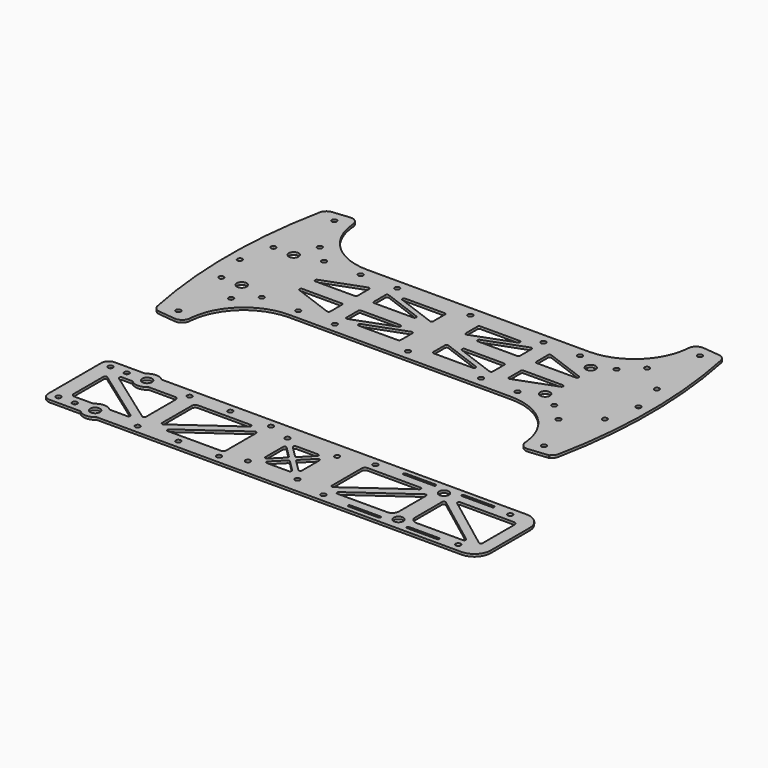
from build123d import *

# Parameters (mm, degrees)
F0_R     = 1.5
F0_R_2   = 3
F1_DEPTH = 1.5
F2_R     = 1.5
F2_R_2   = 3
F3_DEPTH = 1.5


# Not quite as in the source:
# - a feature names something its author has since deleted; it is built from what else it names


with BuildPart() as f1:
    # F0 (on Top) → F1 (new body)
    with BuildSketch(Plane.XY):
        with BuildLine():
            Line((-10.5759569506, 734.1457370259), (-10.5759569506, 711.6457370259))
            Line((-10.5759569506, 711.6457370259), (110.6037002983, 711.6457370259))
            ThreePointArc((110.6037002983, 711.6457370259), (111.0430401265, 712.7063971977), (112.1037002983, 713.1457370259))
            Line((112.1037002983, 713.1457370259), (112.1037002983, 770.2342530502))
            ThreePointArc((112.1037002983, 770.2342530502), (110.7977795433, 768.9107159859), (109.0985539885, 768.1558571299))
            Line((109.0985539885, 768.1558571299), (105.8289895135, 737.0480291089))
            Line((105.8289895135, 737.0480291089), (90.911161083, 738.6159560579))
            Line((90.911161083, 738.6159560579), (91.6428602959, 745.5776090401))
            Line((91.6428602959, 745.5776090401), (95.0922996137, 778.3968318726))
            ThreePointArc((95.0922996137, 778.3968318726), (93.4438470699, 776.7964429634), (92.6851419699, 774.6278012177))
            Line((92.6851419699, 774.6278012177), (92.512712123, 772.9872408115))
            ThreePointArc((92.512712123, 772.9872408115), (81.1240170077, 750.6356681342), (57.7044457851, 741.6457370259))
            Line((57.7044457851, 741.6457370259), (-10.5759569506, 741.6457370259))
            Line((-10.5759569506, 741.6457370259), (-10.5759569506, 737.1457370259))
            ThreePointArc((-10.5759569506, 737.1457370259), (-9.5152967788, 736.7063971977), (-9.0759569506, 735.6457370259))
            ThreePointArc((-9.0759569506, 735.6457370259), (-9.5152967788, 734.5850768541), (-10.5759569506, 734.1457370259))
        make_face()
        Polygon((3.73207875, 716.6457370259), (-0.5759569506, 716.6457370259), (-0.5759569506, 718.2458645718), (-0.5759569506, 719.6840448406), (-0.5759569506, 728.6457370259), (-0.5759569506, 729.6457370259), (0.4240430494, 729.6457370259), (24.5516758561, 729.6457370259), (30.1160073488, 729.6457370259), (34.4240430494, 729.6457370259), (34.4240430494, 728.04560948), (34.4240430494, 726.6074292112), (34.4240430494, 717.6457370259), (34.4240430494, 716.6457370259), (33.4240430494, 716.6457370259), (9.2964102427, 716.6457370259), align=None, mode=Mode.SUBTRACT)
        with Locations((34.4240430494, 735.6457370259)):
            Circle(F0_R, mode=Mode.SUBTRACT)
        with BuildLine():
            Line((79.4240430494, 716.6457370259), (75.1160073488, 716.6457370259))
            Line((75.1160073488, 716.6457370259), (69.5516758561, 716.6457370259))
            Line((69.5516758561, 716.6457370259), (45.4240430494, 716.6457370259))
            Line((45.4240430494, 716.6457370259), (44.4240430494, 716.6457370259))
            Line((44.4240430494, 716.6457370259), (44.4240430494, 717.6457370259))
            Line((44.4240430494, 717.6457370259), (44.4240430494, 726.6074292112))
            Line((44.4240430494, 726.6074292112), (44.4240430494, 728.04560948))
            Line((44.4240430494, 728.04560948), (44.4240430494, 729.6457370259))
            Line((44.4240430494, 729.6457370259), (48.73207875, 729.6457370259))
            Line((48.73207875, 729.6457370259), (54.2964102427, 729.6457370259))
            Line((54.2964102427, 729.6457370259), (65.7160031578, 729.6457370259))
            ThreePointArc((65.7160031578, 729.6457370259), (68.6740430494, 732.1457370259), (71.6320829409, 729.6457370259))
            Line((71.6320829409, 729.6457370259), (78.4240430494, 729.6457370259))
            Line((78.4240430494, 729.6457370259), (79.4240430494, 729.6457370259))
            Line((79.4240430494, 729.6457370259), (79.4240430494, 728.6457370259))
            Line((79.4240430494, 728.6457370259), (79.4240430494, 719.6840448406))
            Line((79.4240430494, 719.6840448406), (79.4240430494, 718.2458645718))
            Line((79.4240430494, 718.2458645718), (79.4240430494, 716.6457370259))
        make_face(mode=Mode.SUBTRACT)
        with Locations((56.9240430494, 735.6457370259)):
            Circle(F0_R, mode=Mode.SUBTRACT)
        with Locations((79.4240430494, 735.6457370259)):
            Circle(F0_R, mode=Mode.SUBTRACT)
        with Locations((107.4240430494, 731.6457370259)):
            Circle(F0_R, mode=Mode.SUBTRACT)
        with BuildLine():
            ThreePointArc((91.6510774828, 745.7344020204), (91.6490217775, 745.6558979427), (91.6428602959, 745.5776090401))
            ThreePointArc((91.6428602959, 745.5776090401), (88.6531331882, 745.812906098), (91.6510774828, 745.7344020204))
        make_face(mode=Mode.SUBTRACT)
        with BuildLine():
            ThreePointArc((-133.2556141995, 713.1457370259), (-132.1949540277, 712.7063971977), (-131.7556141995, 711.6457370259))
            Line((-131.7556141995, 711.6457370259), (-10.5759569506, 711.6457370259))
            Line((-10.5759569506, 711.6457370259), (-10.5759569506, 734.1457370259))
            ThreePointArc((-10.5759569506, 734.1457370259), (-12.0759569506, 735.6457370259), (-10.5759569506, 737.1457370259))
            Line((-10.5759569506, 737.1457370259), (-10.5759569506, 741.6457370259))
            Line((-10.5759569506, 741.6457370259), (-78.8563596864, 741.6457370259))
            ThreePointArc((-78.8563596864, 741.6457370259), (-102.2759309089, 750.6356681342), (-113.6646260243, 772.9872408115))
            Line((-113.6646260243, 772.9872408115), (-113.8370558712, 774.6278012177))
            ThreePointArc((-113.8370558712, 774.6278012177), (-114.5957609711, 776.7964429634), (-116.244213515, 778.3968318726))
            Line((-116.244213515, 778.3968318726), (-112.7947742123, 745.5776091847))
            Line((-112.7947742123, 745.5776091847), (-112.0630749843, 738.6159560579))
            Line((-112.0630749843, 738.6159560579), (-126.9809034148, 737.0480291089))
            Line((-126.9809034148, 737.0480291089), (-130.2504678897, 768.1558571299))
            ThreePointArc((-130.2504678897, 768.1558571299), (-131.9496934446, 768.9107159859), (-133.2556141995, 770.2342530502))
            Line((-133.2556141995, 770.2342530502), (-133.2556141995, 713.1457370259))
        make_face()
        Polygon((-90.7035897573, 716.6457370259), (-96.26792125, 716.6457370259), (-100.5759569506, 716.6457370259), (-100.5759569506, 718.2458645718), (-100.5759569506, 719.6840448406), (-100.5759569506, 728.6457370259), (-100.5759569506, 729.6457370259), (-99.5759569506, 729.6457370259), (-75.4483241439, 729.6457370259), (-69.8839926512, 729.6457370259), (-65.5759569506, 729.6457370259), (-65.5759569506, 728.04560948), (-65.5759569506, 726.6074292112), (-65.5759569506, 717.6457370259), (-65.5759569506, 716.6457370259), (-66.5759569506, 716.6457370259), align=None, mode=Mode.SUBTRACT)
        with Locations((-128.5759569506, 731.6457370259)):
            Circle(F0_R, mode=Mode.SUBTRACT)
        with Locations((-116.0759569506, 731.6457370259)):
            Circle(F0_R_2, mode=Mode.SUBTRACT)
        with Locations((-100.5759569506, 735.6457370259)):
            Circle(F0_R, mode=Mode.SUBTRACT)
        with Locations((-78.0759569506, 735.6457370259)):
            Circle(F0_R, mode=Mode.SUBTRACT)
        Polygon((-20.5759569506, 718.2458645718), (-20.5759569506, 716.6457370259), (-24.8839926512, 716.6457370259), (-30.4483241439, 716.6457370259), (-54.5759569506, 716.6457370259), (-55.5759569506, 716.6457370259), (-55.5759569506, 717.6457370259), (-55.5759569506, 726.6074292112), (-55.5759569506, 728.04560948), (-55.5759569506, 729.6457370259), (-51.26792125, 729.6457370259), (-45.7035897573, 729.6457370259), (-21.5759569506, 729.6457370259), (-20.5759569506, 729.6457370259), (-20.5759569506, 728.6457370259), (-20.5759569506, 719.6840448406), align=None, mode=Mode.SUBTRACT)
        with Locations((-55.5759569506, 735.6457370259)):
            Circle(F0_R, mode=Mode.SUBTRACT)
        with BuildLine():
            ThreePointArc((-109.8029913841, 745.7344020204), (-111.224487379, 744.2364577219), (-112.7947742123, 745.5776091847))
            ThreePointArc((-112.7947742123, 745.5776091847), (-111.3814953891, 747.2323463188), (-109.8029913841, 745.7344020204))
        make_face(mode=Mode.SUBTRACT)
        with BuildLine():
            Line((-10.5759569506, 711.6457370259), (-131.7556141995, 711.6457370259))
            ThreePointArc((-131.7556141995, 711.6457370259), (-132.1949540277, 710.5850768541), (-133.2556141995, 710.1457370259))
            Line((-133.2556141995, 710.1457370259), (-133.2556141995, 653.0572210016))
            ThreePointArc((-133.2556141995, 653.0572210016), (-131.9496934446, 654.3807580659), (-130.2504678897, 655.1356169219))
            Line((-130.2504678897, 655.1356169219), (-126.9809034148, 686.2434449429))
            Line((-126.9809034148, 686.2434449429), (-112.0630749843, 684.6755179939))
            Line((-112.0630749843, 684.6755179939), (-112.7947741962, 677.7138650203))
            Line((-112.7947741962, 677.7138650203), (-116.244213515, 644.8946421792))
            ThreePointArc((-116.244213515, 644.8946421792), (-114.5957609711, 646.4950310884), (-113.8370558712, 648.6636728341))
            Line((-113.8370558712, 648.6636728341), (-113.6646260243, 650.3042332403))
            ThreePointArc((-113.6646260243, 650.3042332403), (-102.2759309089, 672.6558059176), (-78.8563596864, 681.6457370259))
            Line((-78.8563596864, 681.6457370259), (-10.5759569506, 681.6457370259))
            Line((-10.5759569506, 681.6457370259), (-10.5759569506, 686.1457370259))
            ThreePointArc((-10.5759569506, 686.1457370259), (-12.0759569506, 687.6457370259), (-10.5759569506, 689.1457370259))
            Line((-10.5759569506, 689.1457370259), (-10.5759569506, 711.6457370259))
        make_face()
        with BuildLine():
            ThreePointArc((-109.8029913841, 677.5570720314), (-111.381495466, 676.059127737), (-112.7947741962, 677.7138650203))
            ThreePointArc((-112.7947741962, 677.7138650203), (-111.2244873021, 679.0550163258), (-109.8029913841, 677.5570720314))
        make_face(mode=Mode.SUBTRACT)
        with Locations((-128.5759569506, 691.6457370259)):
            Circle(F0_R, mode=Mode.SUBTRACT)
        with Locations((-116.0759569506, 691.6457370259)):
            Circle(F0_R_2, mode=Mode.SUBTRACT)
        with Locations((-100.5759569506, 687.6457370259)):
            Circle(F0_R, mode=Mode.SUBTRACT)
        with Locations((-78.0759569506, 687.6457370259)):
            Circle(F0_R, mode=Mode.SUBTRACT)
        Polygon((-100.5759569506, 706.6457370259), (-96.26792125, 706.6457370259), (-90.7035897573, 706.6457370259), (-66.5759569506, 706.6457370259), (-65.5759569506, 706.6457370259), (-65.5759569506, 705.6457370259), (-65.5759569506, 696.6840448406), (-65.5759569506, 695.2458645718), (-65.5759569506, 693.6457370259), (-69.8839926512, 693.6457370259), (-75.4483241439, 693.6457370259), (-99.5759569506, 693.6457370259), (-100.5759569506, 693.6457370259), (-100.5759569506, 694.6457370259), (-100.5759569506, 703.6074292112), (-100.5759569506, 705.04560948), align=None, mode=Mode.SUBTRACT)
        with Locations((-55.5759569506, 687.6457370259)):
            Circle(F0_R, mode=Mode.SUBTRACT)
        Polygon((-24.8839926512, 706.6457370259), (-20.5759569506, 706.6457370259), (-20.5759569506, 705.04560948), (-20.5759569506, 703.6074292112), (-20.5759569506, 694.6457370259), (-20.5759569506, 693.6457370259), (-21.5759569506, 693.6457370259), (-45.7035897573, 693.6457370259), (-51.26792125, 693.6457370259), (-55.5759569506, 693.6457370259), (-55.5759569506, 695.2458645718), (-55.5759569506, 696.6840448406), (-55.5759569506, 705.6457370259), (-55.5759569506, 706.6457370259), (-54.5759569506, 706.6457370259), (-30.4483241439, 706.6457370259), align=None, mode=Mode.SUBTRACT)
        with BuildLine():
            Line((110.6037002983, 711.6457370259), (-10.5759569506, 711.6457370259))
            Line((-10.5759569506, 711.6457370259), (-10.5759569506, 689.1457370259))
            ThreePointArc((-10.5759569506, 689.1457370259), (-9.5152967788, 688.7063971977), (-9.0759569506, 687.6457370259))
            ThreePointArc((-9.0759569506, 687.6457370259), (-9.5152967788, 686.5850768541), (-10.5759569506, 686.1457370259))
            Line((-10.5759569506, 686.1457370259), (-10.5759569506, 681.6457370259))
            Line((-10.5759569506, 681.6457370259), (57.7044457851, 681.6457370259))
            ThreePointArc((57.7044457851, 681.6457370259), (81.1240170077, 672.6558059176), (92.512712123, 650.3042332403))
            Line((92.512712123, 650.3042332403), (92.6851419699, 648.6636728341))
            ThreePointArc((92.6851419699, 648.6636728341), (93.4438470699, 646.4950310884), (95.0922996137, 644.8946421792))
            Line((95.0922996137, 644.8946421792), (91.6428603111, 677.7138648671))
            Line((91.6428603111, 677.7138648671), (90.911161083, 684.6755179939))
            Line((90.911161083, 684.6755179939), (105.8289895135, 686.2434449429))
            Line((105.8289895135, 686.2434449429), (109.0985539885, 655.1356169219))
            ThreePointArc((109.0985539885, 655.1356169219), (110.7977795433, 654.3807580659), (112.1037002983, 653.0572210016))
            Line((112.1037002983, 653.0572210016), (112.1037002983, 710.1457370259))
            ThreePointArc((112.1037002983, 710.1457370259), (111.0430401265, 710.5850768541), (110.6037002983, 711.6457370259))
        make_face()
        with BuildLine():
            ThreePointArc((91.6510774828, 677.5570720314), (88.6531331844, 677.4785680264), (91.6428603111, 677.7138648671))
            ThreePointArc((91.6428603111, 677.7138648671), (91.6490217813, 677.6355760365), (91.6510774828, 677.5570720314))
        make_face(mode=Mode.SUBTRACT)
        with Locations((34.4240430494, 687.6457370259)):
            Circle(F0_R, mode=Mode.SUBTRACT)
        Polygon((-0.5759569506, 705.04560948), (-0.5759569506, 706.6457370259), (3.73207875, 706.6457370259), (9.2964102427, 706.6457370259), (33.4240430494, 706.6457370259), (34.4240430494, 706.6457370259), (34.4240430494, 705.6457370259), (34.4240430494, 696.6840448406), (34.4240430494, 695.2458645718), (34.4240430494, 693.6457370259), (30.1160073488, 693.6457370259), (24.5516758561, 693.6457370259), (0.4240430494, 693.6457370259), (-0.5759569506, 693.6457370259), (-0.5759569506, 694.6457370259), (-0.5759569506, 703.6074292112), align=None, mode=Mode.SUBTRACT)
        with Locations((56.9240430494, 687.6457370259)):
            Circle(F0_R, mode=Mode.SUBTRACT)
        with Locations((79.4240430494, 687.6457370259)):
            Circle(F0_R, mode=Mode.SUBTRACT)
        with Locations((107.4240430494, 691.6457370259)):
            Circle(F0_R, mode=Mode.SUBTRACT)
        with BuildLine():
            Line((75.1160073488, 706.6457370259), (79.4240430494, 706.6457370259))
            Line((79.4240430494, 706.6457370259), (79.4240430494, 705.04560948))
            Line((79.4240430494, 705.04560948), (79.4240430494, 703.6074292112))
            Line((79.4240430494, 703.6074292112), (79.4240430494, 694.6457370259))
            Line((79.4240430494, 694.6457370259), (79.4240430494, 693.6457370259))
            Line((79.4240430494, 693.6457370259), (78.4240430494, 693.6457370259))
            Line((78.4240430494, 693.6457370259), (71.6320829409, 693.6457370259))
            ThreePointArc((71.6320829409, 693.6457370259), (68.6740430494, 691.1457370259), (65.7160031578, 693.6457370259))
            Line((65.7160031578, 693.6457370259), (54.2964102427, 693.6457370259))
            Line((54.2964102427, 693.6457370259), (48.73207875, 693.6457370259))
            Line((48.73207875, 693.6457370259), (44.4240430494, 693.6457370259))
            Line((44.4240430494, 693.6457370259), (44.4240430494, 695.2458645718))
            Line((44.4240430494, 695.2458645718), (44.4240430494, 696.6840448406))
            Line((44.4240430494, 696.6840448406), (44.4240430494, 705.6457370259))
            Line((44.4240430494, 705.6457370259), (44.4240430494, 706.6457370259))
            Line((44.4240430494, 706.6457370259), (45.4240430494, 706.6457370259))
            Line((45.4240430494, 706.6457370259), (69.5516758561, 706.6457370259))
            Line((69.5516758561, 706.6457370259), (75.1160073488, 706.6457370259))
        make_face(mode=Mode.SUBTRACT)
        with BuildLine():
            ThreePointArc((-133.2556141995, 710.1457370259), (-134.7556141995, 711.6457370259), (-133.2556141995, 713.1457370259))
            Line((-133.2556141995, 713.1457370259), (-133.2556141995, 770.2342530502))
            ThreePointArc((-133.2556141995, 770.2342530502), (-134.009872948, 772.0494219687), (-134.0061738765, 774.0150594682))
            ThreePointArc((-134.0061738765, 774.0150594682), (-140.2556141995, 711.6457372679), (-134.0061739725, 649.2764150579))
            ThreePointArc((-134.0061739725, 649.2764150579), (-134.0098729009, 651.2420523204), (-133.2556141995, 653.0572210016))
            Line((-133.2556141995, 653.0572210016), (-133.2556141995, 710.1457370259))
        make_face()
        with BuildLine():
            Line((112.1037002983, 770.2342530502), (112.1037002983, 713.1457370259))
            ThreePointArc((112.1037002983, 713.1457370259), (113.16436047, 712.7063971977), (113.6037002983, 711.6457370259))
            ThreePointArc((113.6037002983, 711.6457370259), (113.16436047, 710.5850768541), (112.1037002983, 710.1457370259))
            Line((112.1037002983, 710.1457370259), (112.1037002983, 653.0572210016))
            ThreePointArc((112.1037002983, 653.0572210016), (112.7364545933, 651.7261653479), (112.9536633084, 650.268459093))
            ThreePointArc((112.9536633084, 650.268459093), (112.9287504204, 649.769953097), (112.8542600171, 649.2764147905))
            ThreePointArc((112.8542600171, 649.2764147905), (119.1037002983, 711.64573688), (112.854260075, 774.0150589753))
            ThreePointArc((112.854260075, 774.0150589753), (112.9287504349, 773.5215208097), (112.9536633084, 773.0230149588))
            ThreePointArc((112.9536633084, 773.0230149588), (112.7364545933, 771.5653087039), (112.1037002983, 770.2342530502))
        make_face()
        with BuildLine():
            ThreePointArc((-124.4813192926, 771.1213739), (-126.8197356751, 768.5761139615), (-130.2504678897, 768.1558571299))
            Line((-130.2504678897, 768.1558571299), (-126.9809034148, 737.0480291089))
            Line((-126.9809034148, 737.0480291089), (-112.0630749843, 738.6159560579))
            Line((-112.0630749843, 738.6159560579), (-112.7947742123, 745.5776091847))
            Line((-112.7947742123, 745.5776091847), (-116.244213515, 778.3968318726))
            ThreePointArc((-116.244213515, 778.3968318726), (-117.7330101982, 778.9878644719), (-119.3323076643, 779.0777683782))
            Line((-119.3323076643, 779.0777683782), (-129.6282194859, 777.9956244398))
            ThreePointArc((-129.6282194859, 777.9956244398), (-125.7599241629, 776.7387390727), (-124.1055772096, 773.0230149588))
            ThreePointArc((-124.1055772096, 773.0230149588), (-124.1077512655, 772.8755841871), (-124.1142715426, 772.7282816246))
            ThreePointArc((-124.1142715426, 772.7282816246), (-122.4875148923, 773.0254964049), (-121.5759569506, 771.6457370259))
            ThreePointArc((-121.5759569506, 771.6457370259), (-122.8095395271, 770.1695860321), (-124.4813192926, 771.1213739))
        make_face()
        with BuildLine():
            Line((-117.3492698509, 741.0768794277), (-122.3218793277, 740.5542371113))
            ThreePointArc((-122.3218793277, 740.5542371113), (-123.7895770364, 740.9889889791), (-124.519980045, 742.3342239755))
            Line((-124.519980045, 742.3342239755), (-126.4537566155, 760.7328790398))
            ThreePointArc((-126.4537566155, 760.7328790398), (-126.0190047476, 762.2005767485), (-124.6737697513, 762.9309797571))
            Line((-124.6737697513, 762.9309797571), (-119.7011602744, 763.4536220734))
            ThreePointArc((-119.7011602744, 763.4536220734), (-118.2334625658, 763.0188702056), (-117.5030595572, 761.6736352092))
            Line((-117.5030595572, 761.6736352092), (-115.5692829867, 743.2749801449))
            ThreePointArc((-115.5692829867, 743.2749801449), (-116.0040348545, 741.8072824363), (-117.3492698509, 741.0768794277))
        make_face(mode=Mode.SUBTRACT)
        with BuildLine():
            Line((-126.9809034148, 686.2434449429), (-130.2504678897, 655.1356169219))
            ThreePointArc((-130.2504678897, 655.1356169219), (-126.8197356751, 654.7153600903), (-124.4813192926, 652.1701001518))
            ThreePointArc((-124.4813192926, 652.1701001518), (-122.8095395271, 653.1218880197), (-121.5759569506, 651.6457370259))
            ThreePointArc((-121.5759569506, 651.6457370259), (-122.4875148923, 650.2659776469), (-124.1142715426, 650.5631924272))
            ThreePointArc((-124.1142715426, 650.5631924272), (-124.1077512655, 650.4158898647), (-124.1055772096, 650.268459093))
            ThreePointArc((-124.1055772096, 650.268459093), (-125.7599240194, 646.5527351083), (-129.6282191018, 645.2958495716))
            Line((-129.6282191018, 645.2958495716), (-119.3323076643, 644.2137056736))
            ThreePointArc((-119.3323076643, 644.2137056736), (-117.7330101982, 644.3036095799), (-116.244213515, 644.8946421792))
            Line((-116.244213515, 644.8946421792), (-112.7947741962, 677.7138650203))
            Line((-112.7947741962, 677.7138650203), (-112.0630749843, 684.6755179939))
            Line((-112.0630749843, 684.6755179939), (-126.9809034148, 686.2434449429))
        make_face()
        with BuildLine():
            ThreePointArc((-124.519980045, 680.9572500763), (-123.7895770364, 682.3024850727), (-122.3218793277, 682.7372369405))
            Line((-122.3218793277, 682.7372369405), (-117.3492698509, 682.2145946241))
            ThreePointArc((-117.3492698509, 682.2145946241), (-116.0040348545, 681.4841916155), (-115.5692829867, 680.0164939069))
            Line((-115.5692829867, 680.0164939069), (-117.5030595572, 661.6178388426))
            ThreePointArc((-117.5030595572, 661.6178388426), (-118.2334625658, 660.2726038462), (-119.7011602744, 659.8378519784))
            Line((-119.7011602744, 659.8378519784), (-124.6737697513, 660.3604942947))
            ThreePointArc((-124.6737697513, 660.3604942947), (-126.0190047476, 661.0908973033), (-126.4537566155, 662.558595012))
            Line((-126.4537566155, 662.558595012), (-124.519980045, 680.9572500763))
        make_face(mode=Mode.SUBTRACT)
        with BuildLine():
            ThreePointArc((103.3294053913, 652.1701001518), (105.6678217739, 654.7153600903), (109.0985539885, 655.1356169219))
            Line((109.0985539885, 655.1356169219), (105.8289895135, 686.2434449429))
            Line((105.8289895135, 686.2434449429), (90.911161083, 684.6755179939))
            Line((90.911161083, 684.6755179939), (91.6428603111, 677.7138648671))
            Line((91.6428603111, 677.7138648671), (95.0922996137, 644.8946421792))
            ThreePointArc((95.0922996137, 644.8946421792), (96.581096297, 644.3036095799), (98.1803937631, 644.2137056736))
            Line((98.1803937631, 644.2137056736), (108.4763080707, 645.2958498733))
            ThreePointArc((108.4763080707, 645.2958498733), (104.4999034781, 646.6530001962), (102.9623576414, 650.5631924272))
            ThreePointArc((102.9623576414, 650.5631924272), (100.4617067857, 651.9797619528), (103.3294053913, 652.1701001518))
        make_face()
        with BuildLine():
            Line((96.1973559497, 682.2145946241), (101.1699654265, 682.7372369405))
            ThreePointArc((101.1699654265, 682.7372369405), (102.6376631351, 682.3024850727), (103.3680661438, 680.9572500763))
            Line((103.3680661438, 680.9572500763), (105.3018427142, 662.558595012))
            ThreePointArc((105.3018427142, 662.558595012), (104.8670908464, 661.0908973033), (103.52185585, 660.3604942947))
            Line((103.52185585, 660.3604942947), (98.5492463732, 659.8378519784))
            ThreePointArc((98.5492463732, 659.8378519784), (97.0815486645, 660.2726038462), (96.3511456559, 661.6178388426))
            Line((96.3511456559, 661.6178388426), (94.4173690855, 680.0164939069))
            ThreePointArc((94.4173690855, 680.0164939069), (94.8521209533, 681.4841916155), (96.1973559497, 682.2145946241))
        make_face(mode=Mode.SUBTRACT)
        with BuildLine():
            Line((105.8289895135, 737.0480291089), (109.0985539885, 768.1558571299))
            ThreePointArc((109.0985539885, 768.1558571299), (105.6678217739, 768.5761139615), (103.3294053913, 771.1213739))
            ThreePointArc((103.3294053913, 771.1213739), (100.4617067857, 771.311712099), (102.9623576414, 772.7282816246))
            ThreePointArc((102.9623576414, 772.7282816246), (104.4999035314, 776.6384739065), (108.4763082175, 777.9956241631))
            Line((108.4763082175, 777.9956241631), (98.1803937631, 779.0777683782))
            ThreePointArc((98.1803937631, 779.0777683782), (96.581096297, 778.9878644719), (95.0922996137, 778.3968318726))
            Line((95.0922996137, 778.3968318726), (91.6428602959, 745.5776090401))
            Line((91.6428602959, 745.5776090401), (90.911161083, 738.6159560579))
            Line((90.911161083, 738.6159560579), (105.8289895135, 737.0480291089))
        make_face()
        with BuildLine():
            ThreePointArc((103.3680661438, 742.3342239755), (102.6376631351, 740.9889889791), (101.1699654265, 740.5542371113))
            Line((101.1699654265, 740.5542371113), (96.1973559497, 741.0768794277))
            ThreePointArc((96.1973559497, 741.0768794277), (94.8521209533, 741.8072824363), (94.4173690855, 743.2749801449))
            Line((94.4173690855, 743.2749801449), (96.3511456559, 761.6736352092))
            ThreePointArc((96.3511456559, 761.6736352092), (97.0815486645, 763.0188702056), (98.5492463732, 763.4536220734))
            Line((98.5492463732, 763.4536220734), (103.52185585, 762.9309797571))
            ThreePointArc((103.52185585, 762.9309797571), (104.8670908464, 762.2005767485), (105.3018427142, 760.7328790398))
            Line((105.3018427142, 760.7328790398), (103.3680661438, 742.3342239755))
        make_face(mode=Mode.SUBTRACT)
        with BuildLine():
            ThreePointArc((-124.519980045, 742.3342239755), (-123.7895770364, 740.9889889791), (-122.3218793277, 740.5542371113))
            Line((-122.3218793277, 740.5542371113), (-117.3492698509, 741.0768794277))
            ThreePointArc((-117.3492698509, 741.0768794277), (-116.0040348545, 741.8072824363), (-115.5692829867, 743.2749801449))
            Line((-115.5692829867, 743.2749801449), (-117.5030595572, 761.6736352092))
            ThreePointArc((-117.5030595572, 761.6736352092), (-118.2334625658, 763.0188702056), (-119.7011602744, 763.4536220734))
            Line((-119.7011602744, 763.4536220734), (-124.6737697513, 762.9309797571))
            ThreePointArc((-124.6737697513, 762.9309797571), (-126.0190047476, 762.2005767485), (-126.4537566155, 760.7328790398))
            Line((-126.4537566155, 760.7328790398), (-124.519980045, 742.3342239755))
        make_face()
        with BuildLine():
            Line((-117.3492698509, 682.2145946241), (-122.3218793277, 682.7372369405))
            ThreePointArc((-122.3218793277, 682.7372369405), (-123.7895770364, 682.3024850727), (-124.519980045, 680.9572500763))
            Line((-124.519980045, 680.9572500763), (-126.4537566155, 662.558595012))
            ThreePointArc((-126.4537566155, 662.558595012), (-126.0190047476, 661.0908973033), (-124.6737697513, 660.3604942947))
            Line((-124.6737697513, 660.3604942947), (-119.7011602744, 659.8378519784))
            ThreePointArc((-119.7011602744, 659.8378519784), (-118.2334625658, 660.2726038462), (-117.5030595572, 661.6178388426))
            Line((-117.5030595572, 661.6178388426), (-115.5692829867, 680.0164939069))
            ThreePointArc((-115.5692829867, 680.0164939069), (-116.0040348545, 681.4841916155), (-117.3492698509, 682.2145946241))
        make_face()
        with BuildLine():
            ThreePointArc((103.3680661438, 680.9572500763), (102.6376631351, 682.3024850727), (101.1699654265, 682.7372369405))
            Line((101.1699654265, 682.7372369405), (96.1973559497, 682.2145946241))
            ThreePointArc((96.1973559497, 682.2145946241), (94.8521209533, 681.4841916155), (94.4173690855, 680.0164939069))
            Line((94.4173690855, 680.0164939069), (96.3511456559, 661.6178388426))
            ThreePointArc((96.3511456559, 661.6178388426), (97.0815486645, 660.2726038462), (98.5492463732, 659.8378519784))
            Line((98.5492463732, 659.8378519784), (103.52185585, 660.3604942947))
            ThreePointArc((103.52185585, 660.3604942947), (104.8670908464, 661.0908973033), (105.3018427142, 662.558595012))
            Line((105.3018427142, 662.558595012), (103.3680661438, 680.9572500763))
        make_face()
        with BuildLine():
            Line((96.1973559497, 741.0768794277), (101.1699654265, 740.5542371113))
            ThreePointArc((101.1699654265, 740.5542371113), (102.6376631351, 740.9889889791), (103.3680661438, 742.3342239755))
            Line((103.3680661438, 742.3342239755), (105.3018427142, 760.7328790398))
            ThreePointArc((105.3018427142, 760.7328790398), (104.8670908464, 762.2005767485), (103.52185585, 762.9309797571))
            Line((103.52185585, 762.9309797571), (98.5492463732, 763.4536220734))
            ThreePointArc((98.5492463732, 763.4536220734), (97.0815486645, 763.0188702056), (96.3511456559, 761.6736352092))
            Line((96.3511456559, 761.6736352092), (94.4173690855, 743.2749801449))
            ThreePointArc((94.4173690855, 743.2749801449), (94.8521209533, 741.8072824363), (96.1973559497, 741.0768794277))
        make_face()
        with BuildLine():
            Line((-100.5759569506, 728.6457370259), (-100.5759569506, 719.6840448406))
            ThreePointArc((-100.5759569506, 719.6840448406), (-99.5759569506, 720.6840448406), (-98.5759569506, 719.6840448406))
            ThreePointArc((-98.5759569506, 719.6840448406), (-98.7549252125, 719.1131622914), (-99.2277707206, 718.7466194573))
            Line((-99.2277707206, 718.7466194573), (-75.1001375828, 727.7083117656))
            ThreePointArc((-75.1001375828, 727.7083117656), (-76.4325561441, 728.4688546643), (-75.4483241439, 729.6457370259))
            Line((-75.4483241439, 729.6457370259), (-99.5759569506, 729.6457370259))
            ThreePointArc((-99.5759569506, 729.6457370259), (-98.8688501694, 729.3528438071), (-98.5759569506, 728.6457370259))
            ThreePointArc((-98.5759569506, 728.6457370259), (-99.5759569506, 727.6457370259), (-100.5759569506, 728.6457370259))
        make_face()
        with BuildLine():
            ThreePointArc((-98.5759569506, 703.6074292112), (-99.5759569506, 702.6074292112), (-100.5759569506, 703.6074292112))
            Line((-100.5759569506, 703.6074292112), (-100.5759569506, 694.6457370259))
            ThreePointArc((-100.5759569506, 694.6457370259), (-99.5759569506, 695.6457370259), (-98.5759569506, 694.6457370259))
            ThreePointArc((-98.5759569506, 694.6457370259), (-98.8688501694, 693.9386302447), (-99.5759569506, 693.6457370259))
            Line((-99.5759569506, 693.6457370259), (-75.4483241439, 693.6457370259))
            ThreePointArc((-75.4483241439, 693.6457370259), (-76.4325561422, 694.822619398), (-75.1001375629, 695.5831622788))
            Line((-75.1001375629, 695.5831622788), (-99.2277707206, 704.5448545945))
            ThreePointArc((-99.2277707206, 704.5448545945), (-98.7549252125, 704.1783117604), (-98.5759569506, 703.6074292112))
        make_face()
        with BuildLine():
            ThreePointArc((78.0758563599, 718.7466196279), (77.8531607014, 720.5050767186), (79.4240430494, 719.6840448406))
            Line((79.4240430494, 719.6840448406), (79.4240430494, 728.6457370259))
            ThreePointArc((79.4240430494, 728.6457370259), (77.7169362682, 727.9386302447), (78.4240430494, 729.6457370259))
            Line((78.4240430494, 729.6457370259), (71.6320829409, 729.6457370259))
            ThreePointArc((71.6320829409, 729.6457370259), (71.6635346177, 729.3966158067), (71.6740430494, 729.1457370259))
            ThreePointArc((71.6740430494, 729.1457370259), (68.4231642685, 726.1562454575), (65.7160031578, 729.6457370259))
            Line((65.7160031578, 729.6457370259), (54.2964102427, 729.6457370259))
            ThreePointArc((54.2964102427, 729.6457370259), (55.0035170239, 729.3528438071), (55.2964102427, 728.6457370259))
            ThreePointArc((55.2964102427, 728.6457370259), (54.8672926019, 727.8247051557), (53.9482235788, 727.7083118038))
            Line((53.9482235788, 727.7083118038), (78.0758563599, 718.7466196279))
        make_face()
        with BuildLine():
            Line((79.4240430494, 694.6457370259), (79.4240430494, 703.6074292112))
            ThreePointArc((79.4240430494, 703.6074292112), (77.8531607014, 702.7863973332), (78.0758563599, 704.5448544239))
            Line((78.0758563599, 704.5448544239), (53.9482239042, 695.5831623689))
            ThreePointArc((53.9482239042, 695.5831623689), (54.8672927444, 695.4667687971), (55.2964102427, 694.6457370259))
            ThreePointArc((55.2964102427, 694.6457370259), (55.0035170239, 693.9386302447), (54.2964102427, 693.6457370259))
            Line((54.2964102427, 693.6457370259), (65.7160031578, 693.6457370259))
            ThreePointArc((65.7160031578, 693.6457370259), (68.4231642685, 697.1352285943), (71.6740430494, 694.1457370259))
            ThreePointArc((71.6740430494, 694.1457370259), (71.6635346177, 693.8948582451), (71.6320829409, 693.6457370259))
            Line((71.6320829409, 693.6457370259), (78.4240430494, 693.6457370259))
            ThreePointArc((78.4240430494, 693.6457370259), (77.7169362682, 695.3528438071), (79.4240430494, 694.6457370259))
        make_face()
        with BuildLine():
            Line((-131.2373882951, 777.5457775543), (-130.2504678897, 768.1558571299))
            ThreePointArc((-130.2504678897, 768.1558571299), (-126.8197356751, 768.5761139615), (-124.4813192926, 771.1213739))
            ThreePointArc((-124.4813192926, 771.1213739), (-124.5382932143, 771.9797619528), (-124.1142715426, 772.7282816246))
            ThreePointArc((-124.1142715426, 772.7282816246), (-124.1077512655, 772.8755841871), (-124.1055772096, 773.0230149588))
            ThreePointArc((-124.1055772096, 773.0230149588), (-125.7599241629, 776.7387390727), (-129.6282194859, 777.9956244398))
            ThreePointArc((-129.6282194859, 777.9956244398), (-130.4517277278, 777.8383943605), (-131.2373882951, 777.5457775543))
        make_face()
        with BuildLine():
            Line((110.0854743939, 645.7456964975), (109.0985539885, 655.1356169219))
            ThreePointArc((109.0985539885, 655.1356169219), (105.6678217739, 654.7153600903), (103.3294053913, 652.1701001518))
            ThreePointArc((103.3294053913, 652.1701001518), (103.4001940432, 651.9121544494), (103.4240430494, 651.6457370259))
            ThreePointArc((103.4240430494, 651.6457370259), (103.3038024284, 651.0572949676), (102.9623576414, 650.5631924272))
            ThreePointArc((102.9623576414, 650.5631924272), (104.4999034781, 646.6530001962), (108.4763080707, 645.2958498733))
            ThreePointArc((108.4763080707, 645.2958498733), (109.2998150303, 645.4530800278), (110.0854743939, 645.7456964975))
        make_face()
        with BuildLine():
            ThreePointArc((103.3294053913, 771.1213739), (105.6678217739, 768.5761139615), (109.0985539885, 768.1558571299))
            Line((109.0985539885, 768.1558571299), (110.0854743939, 777.5457775543))
            ThreePointArc((110.0854743939, 777.5457775543), (109.2998151013, 777.8383940041), (108.4763082175, 777.9956241631))
            ThreePointArc((108.4763082175, 777.9956241631), (104.4999035314, 776.6384739065), (102.9623576414, 772.7282816246))
            ThreePointArc((102.9623576414, 772.7282816246), (103.3038024284, 772.2341790842), (103.4240430494, 771.6457370259))
            ThreePointArc((103.4240430494, 771.6457370259), (103.4001940432, 771.3793196024), (103.3294053913, 771.1213739))
        make_face()
        with BuildLine():
            ThreePointArc((-124.4813192926, 652.1701001518), (-126.8197356751, 654.7153600903), (-130.2504678897, 655.1356169219))
            Line((-130.2504678897, 655.1356169219), (-131.2373882951, 645.7456964975))
            ThreePointArc((-131.2373882951, 645.7456964975), (-130.4517275418, 645.4530796393), (-129.6282191018, 645.2958495716))
            ThreePointArc((-129.6282191018, 645.2958495716), (-125.7599240194, 646.5527351083), (-124.1055772096, 650.268459093))
            ThreePointArc((-124.1055772096, 650.268459093), (-124.1077512655, 650.4158898647), (-124.1142715426, 650.5631924272))
            ThreePointArc((-124.1142715426, 650.5631924272), (-124.5382932143, 651.311712099), (-124.4813192926, 652.1701001518))
        make_face()
        Polygon((-100.5759569506, 716.6457370259), (-96.26792125, 716.6457370259), (-91.0517764468, 718.5831622385), (-66.9241436401, 727.5448544239), (-65.5759569506, 728.04560948), (-65.5759569506, 729.6457370259), align=None)
        Polygon((-100.5759569506, 718.2458645718), (-100.5759569506, 716.6457370259), (-65.5759569506, 729.6457370259), (-69.8839926512, 729.6457370259), (-75.1001375828, 727.7083117656), (-99.2277707206, 718.7466194573), align=None)
        Polygon((-91.0517762713, 704.7083117481), (-96.26792125, 706.6457370259), (-100.5759569506, 706.6457370259), (-65.5759569506, 693.6457370259), (-65.5759569506, 695.2458645718), (-66.9241436401, 695.7466196279), align=None)
        Polygon((-65.5759569506, 693.6457370259), (-100.5759569506, 706.6457370259), (-100.5759569506, 705.04560948), (-99.2277707206, 704.5448545945), (-75.1001375629, 695.5831622788), (-69.8839926512, 693.6457370259), align=None)
        Polygon((-55.5759569506, 693.6457370259), (-20.5759569506, 706.6457370259), (-24.8839926512, 706.6457370259), (-30.1001379809, 704.7083116177), (-54.2277702867, 695.7466196184), (-55.5759569506, 695.2458645718), align=None)
        Polygon((-20.5759569506, 705.04560948), (-20.5759569506, 706.6457370259), (-55.5759569506, 693.6457370259), (-51.26792125, 693.6457370259), (-46.0517763383, 695.5831622788), (-21.9241434646, 704.5448544891), align=None)
        Polygon((-24.8839926512, 716.6457370259), (-20.5759569506, 716.6457370259), (-55.5759569506, 729.6457370259), (-55.5759569506, 728.04560948), (-54.2277701941, 727.544854399), (-30.1001379809, 718.5831624341), align=None)
        Polygon((-55.5759569506, 729.6457370259), (-20.5759569506, 716.6457370259), (-20.5759569506, 718.2458645718), (-21.9241431806, 718.7466194573), (-46.0517764882, 727.7083118287), (-51.26792125, 729.6457370259), align=None)
        Polygon((-0.5759569506, 718.2458645718), (-0.5759569506, 716.6457370259), (34.4240430494, 729.6457370259), (30.1160073488, 729.6457370259), (24.8998625202, 727.7083118038), (0.7722295378, 718.7466195532), align=None)
        Polygon((34.4240430494, 729.6457370259), (-0.5759569506, 716.6457370259), (3.73207875, 716.6457370259), (8.9482240285, 718.5831624151), (33.0758564013, 727.5448544393), (34.4240430494, 728.04560948), align=None)
        Polygon((3.73207875, 706.6457370259), (-0.5759569506, 706.6457370259), (34.4240430494, 693.6457370259), (34.4240430494, 695.2458645718), (33.0758563343, 695.7466196374), (8.9482236142, 704.7083117906), align=None)
        Polygon((34.4240430494, 693.6457370259), (-0.5759569506, 706.6457370259), (-0.5759569506, 705.04560948), (0.7722295536, 704.5448544927), (24.899862169, 695.5831623784), (30.1160073488, 693.6457370259), align=None)
        Polygon((69.8998620861, 718.5831624092), (75.1160073488, 716.6457370259), (79.4240430494, 716.6457370259), (44.4240430494, 729.6457370259), (44.4240430494, 728.04560948), (45.7722297389, 727.5448544239), align=None)
        Polygon((44.4240430494, 729.6457370259), (79.4240430494, 716.6457370259), (79.4240430494, 718.2458645718), (78.0758563599, 718.7466196279), (53.9482235788, 727.7083118038), (48.73207875, 729.6457370259), align=None)
        Polygon((44.4240430494, 693.6457370259), (79.4240430494, 706.6457370259), (75.1160073488, 706.6457370259), (69.8998623701, 704.7083117481), (45.7722297389, 695.7466196279), (44.4240430494, 695.2458645718), align=None)
        Polygon((79.4240430494, 705.04560948), (79.4240430494, 706.6457370259), (44.4240430494, 693.6457370259), (48.73207875, 693.6457370259), (53.9482239042, 695.5831623689), (78.0758563599, 704.5448544239), align=None)
        with BuildLine():
            Line((-133.2556141995, 775.8117768673), (-133.2556141995, 770.2342530502))
            ThreePointArc((-133.2556141995, 770.2342530502), (-131.9496934446, 768.9107159859), (-130.2504678897, 768.1558571299))
            Line((-130.2504678897, 768.1558571299), (-131.2373882951, 777.5457775543))
            ThreePointArc((-131.2373882951, 777.5457775543), (-132.3639653704, 776.8154952282), (-133.2556141995, 775.8117768673))
        make_face()
        with BuildLine():
            Line((112.1037002983, 647.4796971845), (112.1037002983, 653.0572210016))
            ThreePointArc((112.1037002983, 653.0572210016), (110.7977795433, 654.3807580659), (109.0985539885, 655.1356169219))
            Line((109.0985539885, 655.1356169219), (110.0854743939, 645.7456964975))
            ThreePointArc((110.0854743939, 645.7456964975), (111.2120514691, 646.4759788236), (112.1037002983, 647.4796971845))
        make_face()
        with BuildLine():
            ThreePointArc((109.0985539885, 768.1558571299), (110.7977795433, 768.9107159859), (112.1037002983, 770.2342530502))
            Line((112.1037002983, 770.2342530502), (112.1037002983, 775.8117768673))
            ThreePointArc((112.1037002983, 775.8117768673), (111.2120514691, 776.8154952282), (110.0854743939, 777.5457775543))
            Line((110.0854743939, 777.5457775543), (109.0985539885, 768.1558571299))
        make_face()
        with BuildLine():
            ThreePointArc((-130.2504678897, 655.1356169219), (-131.9496934446, 654.3807580659), (-133.2556141995, 653.0572210016))
            Line((-133.2556141995, 653.0572210016), (-133.2556141995, 647.4796971845))
            ThreePointArc((-133.2556141995, 647.4796971845), (-132.3639653704, 646.4759788236), (-131.2373882951, 645.7456964975))
            Line((-131.2373882951, 645.7456964975), (-130.2504678897, 655.1356169219))
        make_face()
        with BuildLine():
            Line((-91.0517764468, 718.5831622385), (-96.26792125, 716.6457370259))
            Line((-96.26792125, 716.6457370259), (-90.7035897573, 716.6457370259))
            ThreePointArc((-90.7035897573, 716.6457370259), (-91.6878217454, 717.4688545969), (-91.0517764468, 718.5831622385))
        make_face()
        with BuildLine():
            Line((-75.1001375828, 727.7083117656), (-69.8839926512, 729.6457370259))
            Line((-69.8839926512, 729.6457370259), (-75.4483241439, 729.6457370259))
            ThreePointArc((-75.4483241439, 729.6457370259), (-74.7412173627, 729.3528438071), (-74.4483241439, 728.6457370259))
            ThreePointArc((-74.4483241439, 728.6457370259), (-74.627292305, 728.0748546217), (-75.1001375828, 727.7083117656))
        make_face()
        with BuildLine():
            Line((-45.7035897573, 729.6457370259), (-51.26792125, 729.6457370259))
            Line((-51.26792125, 729.6457370259), (-46.0517764882, 727.7083118287))
            ThreePointArc((-46.0517764882, 727.7083118287), (-46.6878217415, 728.8226194766), (-45.7035897573, 729.6457370259))
        make_face()
        with BuildLine():
            Line((-30.4483241439, 716.6457370259), (-24.8839926512, 716.6457370259))
            Line((-24.8839926512, 716.6457370259), (-30.1001379809, 718.5831624341))
            ThreePointArc((-30.1001379809, 718.5831624341), (-29.6272924262, 718.2166196045), (-29.4483241439, 717.6457370259))
            ThreePointArc((-29.4483241439, 717.6457370259), (-29.7412173627, 716.9386302447), (-30.4483241439, 716.6457370259))
        make_face()
        with BuildLine():
            Line((8.9482240285, 718.5831624151), (3.73207875, 716.6457370259))
            Line((3.73207875, 716.6457370259), (9.2964102427, 716.6457370259))
            ThreePointArc((9.2964102427, 716.6457370259), (8.3121782098, 717.4688548464), (8.9482240285, 718.5831624151))
        make_face()
        with BuildLine():
            Line((24.8998625202, 727.7083118038), (30.1160073488, 729.6457370259))
            Line((30.1160073488, 729.6457370259), (24.5516758561, 729.6457370259))
            ThreePointArc((24.5516758561, 729.6457370259), (25.2587826373, 729.3528438071), (25.5516758561, 728.6457370259))
            ThreePointArc((25.5516758561, 728.6457370259), (25.3727077264, 728.0748546668), (24.8998625202, 727.7083118038))
        make_face()
        with BuildLine():
            Line((54.2964102427, 729.6457370259), (48.73207875, 729.6457370259))
            Line((48.73207875, 729.6457370259), (53.9482235788, 727.7083118038))
            ThreePointArc((53.9482235788, 727.7083118038), (53.3121782522, 728.8226194415), (54.2964102427, 729.6457370259))
        make_face()
        with BuildLine():
            Line((69.5516758561, 716.6457370259), (75.1160073488, 716.6457370259))
            Line((75.1160073488, 716.6457370259), (69.8998620861, 718.5831624092))
            ThreePointArc((69.8998620861, 718.5831624092), (70.3727075942, 718.2166195751), (70.5516758561, 717.6457370259))
            ThreePointArc((70.5516758561, 717.6457370259), (70.2587826373, 716.9386302447), (69.5516758561, 716.6457370259))
        make_face()
        with BuildLine():
            Line((69.8998623701, 704.7083117481), (75.1160073488, 706.6457370259))
            Line((75.1160073488, 706.6457370259), (69.5516758561, 706.6457370259))
            ThreePointArc((69.5516758561, 706.6457370259), (70.2587826373, 706.3528438071), (70.5516758561, 705.6457370259))
            ThreePointArc((70.5516758561, 705.6457370259), (70.3727076807, 705.074854601), (69.8998623701, 704.7083117481))
        make_face()
        with BuildLine():
            Line((53.9482239042, 695.5831623689), (48.73207875, 693.6457370259))
            Line((48.73207875, 693.6457370259), (54.2964102427, 693.6457370259))
            ThreePointArc((54.2964102427, 693.6457370259), (53.3121782215, 694.4688547812), (53.9482239042, 695.5831623689))
        make_face()
        with BuildLine():
            Line((24.5516758561, 693.6457370259), (30.1160073488, 693.6457370259))
            Line((30.1160073488, 693.6457370259), (24.899862169, 695.5831623784))
            ThreePointArc((24.899862169, 695.5831623784), (25.3727076194, 695.2166195388), (25.5516758561, 694.6457370259))
            ThreePointArc((25.5516758561, 694.6457370259), (25.2587826373, 693.9386302447), (24.5516758561, 693.6457370259))
        make_face()
        with BuildLine():
            Line((9.2964102427, 706.6457370259), (3.73207875, 706.6457370259))
            Line((3.73207875, 706.6457370259), (8.9482236142, 704.7083117906))
            ThreePointArc((8.9482236142, 704.7083117906), (8.3121782489, 705.8226194229), (9.2964102427, 706.6457370259))
        make_face()
        with BuildLine():
            Line((-30.1001379809, 704.7083116177), (-24.8839926512, 706.6457370259))
            Line((-24.8839926512, 706.6457370259), (-30.4483241439, 706.6457370259))
            ThreePointArc((-30.4483241439, 706.6457370259), (-29.7412173627, 706.3528438071), (-29.4483241439, 705.6457370259))
            ThreePointArc((-29.4483241439, 705.6457370259), (-29.6272924262, 705.0748544473), (-30.1001379809, 704.7083116177))
        make_face()
        with BuildLine():
            Line((-46.0517763383, 695.5831622788), (-51.26792125, 693.6457370259))
            Line((-51.26792125, 693.6457370259), (-45.7035897573, 693.6457370259))
            ThreePointArc((-45.7035897573, 693.6457370259), (-46.6878217556, 694.4688546538), (-46.0517763383, 695.5831622788))
        make_face()
        with BuildLine():
            Line((-75.4483241439, 693.6457370259), (-69.8839926512, 693.6457370259))
            Line((-69.8839926512, 693.6457370259), (-75.1001375629, 695.5831622788))
            ThreePointArc((-75.1001375629, 695.5831622788), (-74.6272922989, 695.2166194214), (-74.4483241439, 694.6457370259))
            ThreePointArc((-74.4483241439, 694.6457370259), (-74.7412173627, 693.9386302447), (-75.4483241439, 693.6457370259))
        make_face()
        with BuildLine():
            Line((-90.7035897573, 706.6457370259), (-96.26792125, 706.6457370259))
            Line((-96.26792125, 706.6457370259), (-91.0517762713, 704.7083117481))
            ThreePointArc((-91.0517762713, 704.7083117481), (-91.6878217619, 705.8226193628), (-90.7035897573, 706.6457370259))
        make_face()
        with BuildLine():
            ThreePointArc((-134.0061738765, 774.0150594682), (-134.009872948, 772.0494219687), (-133.2556141995, 770.2342530502))
            Line((-133.2556141995, 770.2342530502), (-133.2556141995, 775.8117768673))
            ThreePointArc((-133.2556141995, 775.8117768673), (-133.7192027634, 774.9503082032), (-134.0061738765, 774.0150594682))
        make_face()
        with BuildLine():
            ThreePointArc((112.9536633084, 650.268459093), (112.7364545933, 651.7261653479), (112.1037002983, 653.0572210016))
            Line((112.1037002983, 653.0572210016), (112.1037002983, 647.4796971845))
            ThreePointArc((112.1037002983, 647.4796971845), (112.5672889028, 648.341165946), (112.8542600171, 649.2764147905))
            ThreePointArc((112.8542600171, 649.2764147905), (112.9287504204, 649.769953097), (112.9536633084, 650.268459093))
        make_face()
        with BuildLine():
            Line((112.1037002983, 775.8117768673), (112.1037002983, 770.2342530502))
            ThreePointArc((112.1037002983, 770.2342530502), (112.7364545933, 771.5653087039), (112.9536633084, 773.0230149588))
            ThreePointArc((112.9536633084, 773.0230149588), (112.9287504349, 773.5215208097), (112.854260075, 774.0150589753))
            ThreePointArc((112.854260075, 774.0150589753), (112.5672889591, 774.9503079711), (112.1037002983, 775.8117768673))
        make_face()
        with BuildLine():
            Line((-133.2556141995, 647.4796971845), (-133.2556141995, 653.0572210016))
            ThreePointArc((-133.2556141995, 653.0572210016), (-134.0098729009, 651.2420523204), (-134.0061739725, 649.2764150579))
            ThreePointArc((-134.0061739725, 649.2764150579), (-133.7192028566, 648.3411660719), (-133.2556141995, 647.4796971845))
        make_face()
        with BuildLine():
            ThreePointArc((55.2964102427, 694.6457370259), (54.8672927444, 695.4667687971), (53.9482239042, 695.5831623689))
            ThreePointArc((53.9482239042, 695.5831623689), (53.3121782215, 694.4688547812), (54.2964102427, 693.6457370259))
            ThreePointArc((54.2964102427, 693.6457370259), (55.0035170239, 693.9386302447), (55.2964102427, 694.6457370259))
        make_face()
        with BuildLine():
            ThreePointArc((78.0758563599, 704.5448544239), (77.8531607014, 702.7863973332), (79.4240430494, 703.6074292112))
            ThreePointArc((79.4240430494, 703.6074292112), (78.9949253974, 704.4284610893), (78.0758563599, 704.5448544239))
        make_face()
        with BuildLine():
            ThreePointArc((78.4240430494, 693.6457370259), (79.1311498306, 693.9386302447), (79.4240430494, 694.6457370259))
            ThreePointArc((79.4240430494, 694.6457370259), (77.7169362682, 695.3528438071), (78.4240430494, 693.6457370259))
        make_face()
        with BuildLine():
            ThreePointArc((78.0758563599, 718.7466196279), (78.9949253974, 718.8630129625), (79.4240430494, 719.6840448406))
            ThreePointArc((79.4240430494, 719.6840448406), (77.8531607014, 720.5050767186), (78.0758563599, 718.7466196279))
        make_face()
        with BuildLine():
            ThreePointArc((78.4240430494, 729.6457370259), (77.7169362682, 727.9386302447), (79.4240430494, 728.6457370259))
            ThreePointArc((79.4240430494, 728.6457370259), (79.1311498306, 729.3528438071), (78.4240430494, 729.6457370259))
        make_face()
        with BuildLine():
            ThreePointArc((54.2964102427, 729.6457370259), (53.3121782522, 728.8226194415), (53.9482235788, 727.7083118038))
            ThreePointArc((53.9482235788, 727.7083118038), (54.8672926019, 727.8247051557), (55.2964102427, 728.6457370259))
            ThreePointArc((55.2964102427, 728.6457370259), (55.0035170239, 729.3528438071), (54.2964102427, 729.6457370259))
        make_face()
        with BuildLine():
            ThreePointArc((-75.4483241439, 729.6457370259), (-76.4325561441, 728.4688546643), (-75.1001375828, 727.7083117656))
            ThreePointArc((-75.1001375828, 727.7083117656), (-74.627292305, 728.0748546217), (-74.4483241439, 728.6457370259))
            ThreePointArc((-74.4483241439, 728.6457370259), (-74.7412173627, 729.3528438071), (-75.4483241439, 729.6457370259))
        make_face()
        with BuildLine():
            ThreePointArc((-99.5759569506, 729.6457370259), (-100.2830637318, 729.3528438071), (-100.5759569506, 728.6457370259))
            ThreePointArc((-100.5759569506, 728.6457370259), (-99.5759569506, 727.6457370259), (-98.5759569506, 728.6457370259))
            ThreePointArc((-98.5759569506, 728.6457370259), (-98.8688501694, 729.3528438071), (-99.5759569506, 729.6457370259))
        make_face()
        with BuildLine():
            ThreePointArc((-99.2277707206, 704.5448545945), (-100.1468394998, 704.4284609494), (-100.5759569506, 703.6074292112))
            ThreePointArc((-100.5759569506, 703.6074292112), (-99.5759569506, 702.6074292112), (-98.5759569506, 703.6074292112))
            ThreePointArc((-98.5759569506, 703.6074292112), (-98.7549252125, 704.1783117604), (-99.2277707206, 704.5448545945))
        make_face()
        with BuildLine():
            ThreePointArc((-98.5759569506, 694.6457370259), (-99.5759569506, 695.6457370259), (-100.5759569506, 694.6457370259))
            ThreePointArc((-100.5759569506, 694.6457370259), (-100.2830637318, 693.9386302447), (-99.5759569506, 693.6457370259))
            ThreePointArc((-99.5759569506, 693.6457370259), (-98.8688501694, 693.9386302447), (-98.5759569506, 694.6457370259))
        make_face()
        with BuildLine():
            ThreePointArc((-74.4483241439, 694.6457370259), (-74.6272922989, 695.2166194214), (-75.1001375629, 695.5831622788))
            ThreePointArc((-75.1001375629, 695.5831622788), (-76.4325561422, 694.822619398), (-75.4483241439, 693.6457370259))
            ThreePointArc((-75.4483241439, 693.6457370259), (-74.7412173627, 693.9386302447), (-74.4483241439, 694.6457370259))
        make_face()
        with BuildLine():
            ThreePointArc((-98.5759569506, 719.6840448406), (-99.5759569506, 720.6840448406), (-100.5759569506, 719.6840448406))
            ThreePointArc((-100.5759569506, 719.6840448406), (-100.1468394998, 718.8630131024), (-99.2277707206, 718.7466194573))
            ThreePointArc((-99.2277707206, 718.7466194573), (-98.7549252125, 719.1131622914), (-98.5759569506, 719.6840448406))
        make_face()
        with BuildLine():
            Line((-100.5759569506, 719.6840448406), (-100.5759569506, 718.2458645718))
            Line((-100.5759569506, 718.2458645718), (-99.2277707206, 718.7466194573))
            ThreePointArc((-99.2277707206, 718.7466194573), (-100.1468394998, 718.8630131024), (-100.5759569506, 719.6840448406))
        make_face()
        with BuildLine():
            Line((-65.5759569506, 728.04560948), (-66.9241436401, 727.5448544239))
            ThreePointArc((-66.9241436401, 727.5448544239), (-66.0050746026, 727.4284610893), (-65.5759569506, 726.6074292112))
            Line((-65.5759569506, 726.6074292112), (-65.5759569506, 728.04560948))
        make_face()
        with BuildLine():
            Line((-54.2277701941, 727.544854399), (-55.5759569506, 728.04560948))
            Line((-55.5759569506, 728.04560948), (-55.5759569506, 726.6074292112))
            ThreePointArc((-55.5759569506, 726.6074292112), (-55.1468392693, 727.4284611097), (-54.2277701941, 727.544854399))
        make_face()
        with BuildLine():
            Line((-21.9241431806, 718.7466194573), (-20.5759569506, 718.2458645718))
            Line((-20.5759569506, 718.2458645718), (-20.5759569506, 719.6840448406))
            ThreePointArc((-20.5759569506, 719.6840448406), (-21.0050744014, 718.8630131024), (-21.9241431806, 718.7466194573))
        make_face()
        with BuildLine():
            Line((-0.5759569506, 719.6840448406), (-0.5759569506, 718.2458645718))
            Line((-0.5759569506, 718.2458645718), (0.7722295378, 718.7466195532))
            ThreePointArc((0.7722295378, 718.7466195532), (-0.1468393867, 718.8630130238), (-0.5759569506, 719.6840448406))
        make_face()
        with BuildLine():
            Line((34.4240430494, 726.6074292112), (34.4240430494, 728.04560948))
            Line((34.4240430494, 728.04560948), (33.0758564013, 727.5448544393))
            ThreePointArc((33.0758564013, 727.5448544393), (33.9949254155, 727.4284610767), (34.4240430494, 726.6074292112))
        make_face()
        with BuildLine():
            ThreePointArc((44.4240430494, 726.6074292112), (44.8531607014, 727.4284610893), (45.7722297389, 727.5448544239))
            Line((45.7722297389, 727.5448544239), (44.4240430494, 728.04560948))
            Line((44.4240430494, 728.04560948), (44.4240430494, 726.6074292112))
        make_face()
        with BuildLine():
            Line((78.0758563599, 718.7466196279), (79.4240430494, 718.2458645718))
            Line((79.4240430494, 718.2458645718), (79.4240430494, 719.6840448406))
            ThreePointArc((79.4240430494, 719.6840448406), (78.9949253974, 718.8630129625), (78.0758563599, 718.7466196279))
        make_face()
        with BuildLine():
            Line((79.4240430494, 703.6074292112), (79.4240430494, 705.04560948))
            Line((79.4240430494, 705.04560948), (78.0758563599, 704.5448544239))
            ThreePointArc((78.0758563599, 704.5448544239), (78.9949253974, 704.4284610893), (79.4240430494, 703.6074292112))
        make_face()
        with BuildLine():
            Line((44.4240430494, 696.6840448406), (44.4240430494, 695.2458645718))
            Line((44.4240430494, 695.2458645718), (45.7722297389, 695.7466196279))
            ThreePointArc((45.7722297389, 695.7466196279), (44.8531607014, 695.8630129625), (44.4240430494, 696.6840448406))
        make_face()
        with BuildLine():
            Line((33.0758563343, 695.7466196374), (34.4240430494, 695.2458645718))
            Line((34.4240430494, 695.2458645718), (34.4240430494, 696.6840448406))
            ThreePointArc((34.4240430494, 696.6840448406), (33.9949253862, 695.8630129547), (33.0758563343, 695.7466196374))
        make_face()
        with BuildLine():
            Line((0.7722295536, 704.5448544927), (-0.5759569506, 705.04560948))
            Line((-0.5759569506, 705.04560948), (-0.5759569506, 703.6074292112))
            ThreePointArc((-0.5759569506, 703.6074292112), (-0.1468393798, 704.4284610329), (0.7722295536, 704.5448544927))
        make_face()
        with BuildLine():
            Line((-20.5759569506, 703.6074292112), (-20.5759569506, 705.04560948))
            Line((-20.5759569506, 705.04560948), (-21.9241434646, 704.5448544891))
            ThreePointArc((-21.9241434646, 704.5448544891), (-21.0050745258, 704.4284610358), (-20.5759569506, 703.6074292112))
        make_face()
        with BuildLine():
            Line((-55.5759569506, 696.6840448406), (-55.5759569506, 695.2458645718))
            Line((-55.5759569506, 695.2458645718), (-54.2277702867, 695.7466196184))
            ThreePointArc((-54.2277702867, 695.7466196184), (-55.1468393098, 695.8630129703), (-55.5759569506, 696.6840448406))
        make_face()
        with BuildLine():
            ThreePointArc((-65.5759569506, 696.6840448406), (-66.0050746026, 695.8630129625), (-66.9241436401, 695.7466196279))
            Line((-66.9241436401, 695.7466196279), (-65.5759569506, 695.2458645718))
            Line((-65.5759569506, 695.2458645718), (-65.5759569506, 696.6840448406))
        make_face()
        with BuildLine():
            Line((-99.2277707206, 704.5448545945), (-100.5759569506, 705.04560948))
            Line((-100.5759569506, 705.04560948), (-100.5759569506, 703.6074292112))
            ThreePointArc((-100.5759569506, 703.6074292112), (-100.1468394998, 704.4284609494), (-99.2277707206, 704.5448545945))
        make_face()
        with BuildLine():
            Line((-100.5759569506, 729.6457370259), (-100.5759569506, 728.6457370259))
            ThreePointArc((-100.5759569506, 728.6457370259), (-100.2830637318, 729.3528438071), (-99.5759569506, 729.6457370259))
            Line((-99.5759569506, 729.6457370259), (-100.5759569506, 729.6457370259))
        make_face()
        with BuildLine():
            ThreePointArc((-65.5759569506, 717.6457370259), (-65.8688501694, 716.9386302447), (-66.5759569506, 716.6457370259))
            Line((-66.5759569506, 716.6457370259), (-65.5759569506, 716.6457370259))
            Line((-65.5759569506, 716.6457370259), (-65.5759569506, 717.6457370259))
        make_face()
        with BuildLine():
            Line((-55.5759569506, 716.6457370259), (-54.5759569506, 716.6457370259))
            ThreePointArc((-54.5759569506, 716.6457370259), (-55.2830637318, 716.9386302447), (-55.5759569506, 717.6457370259))
            Line((-55.5759569506, 717.6457370259), (-55.5759569506, 716.6457370259))
        make_face()
        with BuildLine():
            ThreePointArc((-21.5759569506, 729.6457370259), (-20.8688501694, 729.3528438071), (-20.5759569506, 728.6457370259))
            Line((-20.5759569506, 728.6457370259), (-20.5759569506, 729.6457370259))
            Line((-20.5759569506, 729.6457370259), (-21.5759569506, 729.6457370259))
        make_face()
        with BuildLine():
            Line((-0.5759569506, 729.6457370259), (-0.5759569506, 728.6457370259))
            ThreePointArc((-0.5759569506, 728.6457370259), (-0.2830637318, 729.3528438071), (0.4240430494, 729.6457370259))
            Line((0.4240430494, 729.6457370259), (-0.5759569506, 729.6457370259))
        make_face()
        with BuildLine():
            ThreePointArc((34.4240430494, 717.6457370259), (34.1311498306, 716.9386302447), (33.4240430494, 716.6457370259))
            Line((33.4240430494, 716.6457370259), (34.4240430494, 716.6457370259))
            Line((34.4240430494, 716.6457370259), (34.4240430494, 717.6457370259))
        make_face()
        with BuildLine():
            Line((44.4240430494, 716.6457370259), (45.4240430494, 716.6457370259))
            ThreePointArc((45.4240430494, 716.6457370259), (44.7169362682, 716.9386302447), (44.4240430494, 717.6457370259))
            Line((44.4240430494, 717.6457370259), (44.4240430494, 716.6457370259))
        make_face()
        with BuildLine():
            ThreePointArc((78.4240430494, 729.6457370259), (79.1311498306, 729.3528438071), (79.4240430494, 728.6457370259))
            Line((79.4240430494, 728.6457370259), (79.4240430494, 729.6457370259))
            Line((79.4240430494, 729.6457370259), (78.4240430494, 729.6457370259))
        make_face()
        with BuildLine():
            Line((79.4240430494, 693.6457370259), (79.4240430494, 694.6457370259))
            ThreePointArc((79.4240430494, 694.6457370259), (79.1311498306, 693.9386302447), (78.4240430494, 693.6457370259))
            Line((78.4240430494, 693.6457370259), (79.4240430494, 693.6457370259))
        make_face()
        with BuildLine():
            ThreePointArc((44.4240430494, 705.6457370259), (44.7169362682, 706.3528438071), (45.4240430494, 706.6457370259))
            Line((45.4240430494, 706.6457370259), (44.4240430494, 706.6457370259))
            Line((44.4240430494, 706.6457370259), (44.4240430494, 705.6457370259))
        make_face()
        with BuildLine():
            Line((34.4240430494, 706.6457370259), (33.4240430494, 706.6457370259))
            ThreePointArc((33.4240430494, 706.6457370259), (34.1311498306, 706.3528438071), (34.4240430494, 705.6457370259))
            Line((34.4240430494, 705.6457370259), (34.4240430494, 706.6457370259))
        make_face()
        with BuildLine():
            ThreePointArc((0.4240430494, 693.6457370259), (-0.2830637318, 693.9386302447), (-0.5759569506, 694.6457370259))
            Line((-0.5759569506, 694.6457370259), (-0.5759569506, 693.6457370259))
            Line((-0.5759569506, 693.6457370259), (0.4240430494, 693.6457370259))
        make_face()
        with BuildLine():
            Line((-20.5759569506, 693.6457370259), (-20.5759569506, 694.6457370259))
            ThreePointArc((-20.5759569506, 694.6457370259), (-20.8688501694, 693.9386302447), (-21.5759569506, 693.6457370259))
            Line((-21.5759569506, 693.6457370259), (-20.5759569506, 693.6457370259))
        make_face()
        with BuildLine():
            ThreePointArc((-55.5759569506, 705.6457370259), (-55.2830637318, 706.3528438071), (-54.5759569506, 706.6457370259))
            Line((-54.5759569506, 706.6457370259), (-55.5759569506, 706.6457370259))
            Line((-55.5759569506, 706.6457370259), (-55.5759569506, 705.6457370259))
        make_face()
        with BuildLine():
            Line((-65.5759569506, 706.6457370259), (-66.5759569506, 706.6457370259))
            ThreePointArc((-66.5759569506, 706.6457370259), (-65.8688501694, 706.3528438071), (-65.5759569506, 705.6457370259))
            Line((-65.5759569506, 705.6457370259), (-65.5759569506, 706.6457370259))
        make_face()
        with BuildLine():
            ThreePointArc((-99.5759569506, 693.6457370259), (-100.2830637318, 693.9386302447), (-100.5759569506, 694.6457370259))
            Line((-100.5759569506, 694.6457370259), (-100.5759569506, 693.6457370259))
            Line((-100.5759569506, 693.6457370259), (-99.5759569506, 693.6457370259))
        make_face()
        with BuildLine():
            Line((110.1146565075, 645.4680472328), (110.0854743939, 645.7456964975))
            ThreePointArc((110.0854743939, 645.7456964975), (109.2998150303, 645.4530800278), (108.4763080707, 645.2958498733))
            Line((108.4763080707, 645.2958498733), (110.1146565075, 645.4680472328))
        make_face()
    extrude(amount=F1_DEPTH)


with BuildPart() as f3:
    # F2 (on Top) → F3 (new body)
    with BuildSketch(Plane.XY):
        with BuildLine():
            Line((149.9681245536, 550.6419631958), (149.9681245536, 565.6419631958))
            Line((149.9681245536, 565.6419631958), (142.2181245536, 565.6419631958))
            Line((142.2181245536, 565.6419631958), (142.2181245536, 554.0834925206))
            Line((142.2181245536, 554.0834925206), (142.2181245536, 552.0759396677))
            Line((142.2181245536, 552.0759396677), (142.2181245536, 550.6419631958))
            Line((142.2181245536, 550.6419631958), (139.9681245536, 550.6419631958))
            Line((139.9681245536, 550.6419631958), (135.8181057283, 550.6419631958))
            Line((135.8181057283, 550.6419631958), (132.8330981982, 550.6419631958))
            Line((132.8330981982, 550.6419631958), (104.2181245536, 550.6419631958))
            ThreePointArc((104.2181245536, 550.6419631958), (101.3896974288, 551.8135360711), (100.2181245536, 554.6419631958))
            Line((100.2181245536, 554.6419631958), (100.2181245536, 565.6419631958))
            Line((100.2181245536, 565.6419631958), (90.2181245536, 565.6419631958))
            Line((90.2181245536, 565.6419631958), (90.2181245536, 554.6419631958))
            ThreePointArc((90.2181245536, 554.6419631958), (89.0465516783, 551.8135360711), (86.2181245536, 550.6419631958))
            Line((86.2181245536, 550.6419631958), (55.6397522405, 550.6419631958))
            Line((55.6397522405, 550.6419631958), (52.5192871871, 550.6419631958))
            Line((52.5192871871, 550.6419631958), (48.2181245536, 550.6419631958))
            Line((48.2181245536, 550.6419631958), (48.2181245536, 553.7142222197))
            Line((48.2181245536, 553.7142222197), (48.2181245536, 555.6574115436))
            Line((48.2181245536, 555.6574115436), (48.2181245536, 565.6419631958))
            Line((48.2181245536, 565.6419631958), (31.2181245536, 565.6419631958))
            Line((31.2181245536, 565.6419631958), (31.2181245536, 551.8919631958))
            ThreePointArc((31.2181245536, 551.8919631958), (32.2787847253, 551.4526233676), (32.7181245536, 550.3919631958))
            ThreePointArc((32.7181245536, 550.3919631958), (31.2181245536, 548.8919631958), (29.7181245536, 550.3919631958))
            Line((29.7181245536, 550.3919631958), (2.2181245536, 550.3919631958))
            ThreePointArc((2.2181245536, 550.3919631958), (-0.3425356182, 549.331303024), (0.7181245536, 551.8919631958))
            Line((0.7181245536, 551.8919631958), (0.7181245536, 565.6419631958))
            Line((0.7181245536, 565.6419631958), (-14.2818754464, 565.6419631958))
            Line((-14.2818754464, 565.6419631958), (-14.2818754464, 552.6419631958))
            ThreePointArc((-14.2818754464, 552.6419631958), (-14.8676618841, 551.2277496334), (-16.2818754464, 550.6419631958))
            Line((-16.2818754464, 550.6419631958), (-48.8602477595, 550.6419631958))
            Line((-48.8602477595, 550.6419631958), (-51.9807128129, 550.6419631958))
            Line((-51.9807128129, 550.6419631958), (-56.2818754464, 550.6419631958))
            Line((-56.2818754464, 550.6419631958), (-56.2818754464, 553.7142222197))
            Line((-56.2818754464, 553.7142222197), (-56.2818754464, 555.6574115436))
            Line((-56.2818754464, 555.6574115436), (-56.2818754464, 565.6419631958))
            Line((-56.2818754464, 565.6419631958), (-66.2818754464, 565.6419631958))
            Line((-66.2818754464, 565.6419631958), (-66.2818754464, 555.6574115436))
            Line((-66.2818754464, 555.6574115436), (-66.2818754464, 553.7142222197))
            Line((-66.2818754464, 553.7142222197), (-66.2818754464, 550.6419631958))
            Line((-66.2818754464, 550.6419631958), (-70.58303808, 550.6419631958))
            Line((-70.58303808, 550.6419631958), (-73.7035031334, 550.6419631958))
            Line((-73.7035031334, 550.6419631958), (-84.2403728243, 550.6419631958))
            Line((-84.2403728243, 550.6419631958), (-84.6328959609, 550.6419631958))
            ThreePointArc((-84.6328959609, 550.6419631958), (-83.0784710581, 548.3537101974), (-82.5318754464, 545.6419631958))
            ThreePointArc((-82.5318754464, 545.6419631958), (-83.0784710581, 542.9302161942), (-84.6328959609, 540.6419631958))
            Line((-84.6328959609, 540.6419631958), (-84.2403728243, 540.6419631958))
            Line((-84.2403728243, 540.6419631958), (139.9681245536, 540.6419631958))
            ThreePointArc((139.9681245536, 540.6419631958), (147.0391923654, 543.5708953839), (149.9681245536, 550.6419631958))
        make_face()
        with Locations((-63.2818754464, 545.6419631958)):
            Circle(F2_R, mode=Mode.SUBTRACT)
        with Locations((-38.2818754464, 545.6419631958)):
            Circle(F2_R, mode=Mode.SUBTRACT)
        with Locations((-13.2818754464, 545.6419631958)):
            Circle(F2_R, mode=Mode.SUBTRACT)
        with BuildLine():
            ThreePointArc((86.4681245536, 545.1419631958), (86.9984546395, 544.9222932817), (87.2181245536, 544.3919631958))
            ThreePointArc((87.2181245536, 544.3919631958), (86.9984546395, 543.8616331099), (86.4681245536, 543.6419631958))
            Line((86.4681245536, 543.6419631958), (67.9681245536, 543.6419631958))
            ThreePointArc((67.9681245536, 543.6419631958), (67.4377944677, 543.8616331099), (67.2181245536, 544.3919631958))
            ThreePointArc((67.2181245536, 544.3919631958), (67.4377944677, 544.9222932817), (67.9681245536, 545.1419631958))
            Line((67.9681245536, 545.1419631958), (86.4681245536, 545.1419631958))
        make_face(mode=Mode.SUBTRACT)
        with Locations((15.9681245536, 545.6419631958)):
            Circle(F2_R, mode=Mode.SUBTRACT)
        with Locations((50.9681245536, 545.6419631958)):
            Circle(F2_R, mode=Mode.SUBTRACT)
        with BuildLine():
            ThreePointArc((122.4681245536, 545.1419631958), (122.9984546395, 544.9222932817), (123.2181245536, 544.3919631958))
            ThreePointArc((123.2181245536, 544.3919631958), (122.9984546395, 543.8616331099), (122.4681245536, 543.6419631958))
            Line((122.4681245536, 543.6419631958), (103.9681245536, 543.6419631958))
            ThreePointArc((103.9681245536, 543.6419631958), (103.4377944677, 543.8616331099), (103.2181245536, 544.3919631958))
            ThreePointArc((103.2181245536, 544.3919631958), (103.4377944677, 544.9222932817), (103.9681245536, 545.1419631958))
            Line((103.9681245536, 545.1419631958), (122.4681245536, 545.1419631958))
        make_face(mode=Mode.SUBTRACT)
        with Locations((95.2181245536, 548.1419631958)):
            Circle(F2_R_2, mode=Mode.SUBTRACT)
        with Locations((133.9681245536, 545.6419631958)):
            Circle(F2_R, mode=Mode.SUBTRACT)
        with BuildLine():
            ThreePointArc((149.9681245536, 580.6419631958), (147.0391923654, 587.7130310077), (139.9681245536, 590.6419631958))
            Line((139.9681245536, 590.6419631958), (-84.2403728243, 590.6419631958))
            Line((-84.2403728243, 590.6419631958), (-84.6328959609, 590.6419631958))
            ThreePointArc((-84.6328959609, 590.6419631958), (-83.0784710581, 588.3537101974), (-82.5318754464, 585.6419631958))
            ThreePointArc((-82.5318754464, 585.6419631958), (-83.0784710581, 582.9302161942), (-84.6328959609, 580.6419631958))
            Line((-84.6328959609, 580.6419631958), (-84.2403728243, 580.6419631958))
            Line((-84.2403728243, 580.6419631958), (-68.2818754464, 580.6419631958))
            ThreePointArc((-68.2818754464, 580.6419631958), (-66.8676618841, 580.0561767582), (-66.2818754464, 578.6419631958))
            Line((-66.2818754464, 578.6419631958), (-66.2818754464, 565.6419631958))
            Line((-66.2818754464, 565.6419631958), (-56.2818754464, 565.6419631958))
            Line((-56.2818754464, 565.6419631958), (-56.2818754464, 578.6419631958))
            ThreePointArc((-56.2818754464, 578.6419631958), (-55.6960890088, 580.0561767582), (-54.2818754464, 580.6419631958))
            Line((-54.2818754464, 580.6419631958), (-21.7035031334, 580.6419631958))
            Line((-21.7035031334, 580.6419631958), (-18.58303808, 580.6419631958))
            Line((-18.58303808, 580.6419631958), (-14.2818754464, 580.6419631958))
            Line((-14.2818754464, 580.6419631958), (-14.2818754464, 577.5697041719))
            Line((-14.2818754464, 577.5697041719), (-14.2818754464, 575.626514848))
            Line((-14.2818754464, 575.626514848), (-14.2818754464, 565.6419631958))
            Line((-14.2818754464, 565.6419631958), (0.7181245536, 565.6419631958))
            Line((0.7181245536, 565.6419631958), (0.7181245536, 579.3919631958))
            ThreePointArc((0.7181245536, 579.3919631958), (-0.3425356182, 581.9526233676), (2.2181245536, 580.8919631958))
            Line((2.2181245536, 580.8919631958), (29.7181245536, 580.8919631958))
            ThreePointArc((29.7181245536, 580.8919631958), (31.2181245536, 582.3919631958), (32.7181245536, 580.8919631958))
            ThreePointArc((32.7181245536, 580.8919631958), (32.2787847253, 579.831303024), (31.2181245536, 579.3919631958))
            Line((31.2181245536, 579.3919631958), (31.2181245536, 565.6419631958))
            Line((31.2181245536, 565.6419631958), (48.2181245536, 565.6419631958))
            Line((48.2181245536, 565.6419631958), (48.2181245536, 578.6419631958))
            ThreePointArc((48.2181245536, 578.6419631958), (48.8039109912, 580.0561767582), (50.2181245536, 580.6419631958))
            Line((50.2181245536, 580.6419631958), (82.7964968666, 580.6419631958))
            Line((82.7964968666, 580.6419631958), (85.91696192, 580.6419631958))
            Line((85.91696192, 580.6419631958), (90.2181245536, 580.6419631958))
            Line((90.2181245536, 580.6419631958), (90.2181245536, 577.5697041719))
            Line((90.2181245536, 577.5697041719), (90.2181245536, 575.626514848))
            Line((90.2181245536, 575.626514848), (90.2181245536, 565.6419631958))
            Line((90.2181245536, 565.6419631958), (100.2181245536, 565.6419631958))
            Line((100.2181245536, 565.6419631958), (100.2181245536, 575.5023206635))
            Line((100.2181245536, 575.5023206635), (100.2181245536, 577.5098735164))
            Line((100.2181245536, 577.5098735164), (100.2181245536, 580.6419631958))
            Line((100.2181245536, 580.6419631958), (104.3681433788, 580.6419631958))
            Line((104.3681433788, 580.6419631958), (107.3531509089, 580.6419631958))
            Line((107.3531509089, 580.6419631958), (140.2181245536, 580.6419631958))
            ThreePointArc((140.2181245536, 580.6419631958), (141.6323381159, 580.0561767582), (142.2181245536, 578.6419631958))
            Line((142.2181245536, 578.6419631958), (142.2181245536, 565.6419631958))
            Line((142.2181245536, 565.6419631958), (149.9681245536, 565.6419631958))
            Line((149.9681245536, 565.6419631958), (149.9681245536, 580.6419631958))
        make_face()
        with Locations((-63.2818754464, 585.6419631958)):
            Circle(F2_R, mode=Mode.SUBTRACT)
        with Locations((-38.2818754464, 585.6419631958)):
            Circle(F2_R, mode=Mode.SUBTRACT)
        with Locations((-13.2818754464, 585.6419631958)):
            Circle(F2_R, mode=Mode.SUBTRACT)
        with Locations((15.9681245536, 585.6419631958)):
            Circle(F2_R, mode=Mode.SUBTRACT)
        with Locations((50.9681245536, 585.6419631958)):
            Circle(F2_R, mode=Mode.SUBTRACT)
        with BuildLine():
            ThreePointArc((87.2181245536, 586.8919631958), (86.9984546395, 586.3616331099), (86.4681245536, 586.1419631958))
            Line((86.4681245536, 586.1419631958), (67.9681245536, 586.1419631958))
            ThreePointArc((67.9681245536, 586.1419631958), (67.4377944677, 586.3616331099), (67.2181245536, 586.8919631958))
            ThreePointArc((67.2181245536, 586.8919631958), (67.4377944677, 587.4222932817), (67.9681245536, 587.6419631958))
            Line((67.9681245536, 587.6419631958), (86.4681245536, 587.6419631958))
            ThreePointArc((86.4681245536, 587.6419631958), (86.9984546395, 587.4222932817), (87.2181245536, 586.8919631958))
        make_face(mode=Mode.SUBTRACT)
        with Locations((95.2181245536, 583.1419631958)):
            Circle(F2_R_2, mode=Mode.SUBTRACT)
        with Locations((133.9681245536, 585.6419631958)):
            Circle(F2_R, mode=Mode.SUBTRACT)
        with BuildLine():
            Line((103.9681245536, 587.6419631958), (122.4681245536, 587.6419631958))
            ThreePointArc((122.4681245536, 587.6419631958), (122.9984546395, 587.4222932817), (123.2181245536, 586.8919631958))
            ThreePointArc((123.2181245536, 586.8919631958), (122.9984546395, 586.3616331099), (122.4681245536, 586.1419631958))
            Line((122.4681245536, 586.1419631958), (103.9681245536, 586.1419631958))
            ThreePointArc((103.9681245536, 586.1419631958), (103.4377944677, 586.3616331099), (103.2181245536, 586.8919631958))
            ThreePointArc((103.2181245536, 586.8919631958), (103.4377944677, 587.4222932817), (103.9681245536, 587.6419631958))
        make_face(mode=Mode.SUBTRACT)
        with BuildLine():
            Line((-108.2818754464, 565.6419631958), (-118.0318754464, 565.6419631958))
            Line((-118.0318754464, 565.6419631958), (-118.0318754464, 545.1419631958))
            ThreePointArc((-118.0318754464, 545.1419631958), (-116.7138559618, 541.9599826805), (-113.5318754464, 540.6419631958))
            Line((-113.5318754464, 540.6419631958), (-94.8233780686, 540.6419631958))
            Line((-94.8233780686, 540.6419631958), (-94.430854932, 540.6419631958))
            ThreePointArc((-94.430854932, 540.6419631958), (-96.5318754464, 545.6419631958), (-94.430854932, 550.6419631958))
            Line((-94.430854932, 550.6419631958), (-94.8233780686, 550.6419631958))
            Line((-94.8233780686, 550.6419631958), (-106.2818754464, 550.6419631958))
            ThreePointArc((-106.2818754464, 550.6419631958), (-107.6960890088, 551.2277496334), (-108.2818754464, 552.6419631958))
            Line((-108.2818754464, 552.6419631958), (-108.2818754464, 565.6419631958))
        make_face()
        with Locations((-112.0318754464, 545.6419631958)):
            Circle(F2_R, mode=Mode.SUBTRACT)
        with Locations((-102.0318754464, 545.6419631958)):
            Circle(F2_R, mode=Mode.SUBTRACT)
        with BuildLine():
            ThreePointArc((-94.430854932, 580.6419631958), (-96.5318754464, 585.6419631958), (-94.430854932, 590.6419631958))
            Line((-94.430854932, 590.6419631958), (-94.8233780686, 590.6419631958))
            Line((-94.8233780686, 590.6419631958), (-113.5318754464, 590.6419631958))
            ThreePointArc((-113.5318754464, 590.6419631958), (-116.7138559618, 589.3239437111), (-118.0318754464, 586.1419631958))
            Line((-118.0318754464, 586.1419631958), (-118.0318754464, 565.6419631958))
            Line((-118.0318754464, 565.6419631958), (-108.2818754464, 565.6419631958))
            Line((-108.2818754464, 565.6419631958), (-108.2818754464, 575.626514848))
            Line((-108.2818754464, 575.626514848), (-108.2818754464, 577.5697041719))
            Line((-108.2818754464, 577.5697041719), (-108.2818754464, 580.6419631958))
            Line((-108.2818754464, 580.6419631958), (-103.9807128129, 580.6419631958))
            Line((-103.9807128129, 580.6419631958), (-100.8602477595, 580.6419631958))
            Line((-100.8602477595, 580.6419631958), (-94.8233780686, 580.6419631958))
            Line((-94.8233780686, 580.6419631958), (-94.430854932, 580.6419631958))
        make_face()
        with Locations((-112.0318754464, 585.6419631958)):
            Circle(F2_R, mode=Mode.SUBTRACT)
        with Locations((-102.0318754464, 585.6419631958)):
            Circle(F2_R, mode=Mode.SUBTRACT)
        with BuildLine():
            Line((27.2181245536, 565.6419631958), (31.2181245536, 565.6419631958))
            Line((31.2181245536, 565.6419631958), (31.2181245536, 579.3919631958))
            ThreePointArc((31.2181245536, 579.3919631958), (30.1574643818, 579.831303024), (29.7181245536, 580.8919631958))
            Line((29.7181245536, 580.8919631958), (2.2181245536, 580.8919631958))
            ThreePointArc((2.2181245536, 580.8919631958), (1.7787847253, 579.831303024), (0.7181245536, 579.3919631958))
            Line((0.7181245536, 579.3919631958), (0.7181245536, 565.6419631958))
            Line((0.7181245536, 565.6419631958), (4.7181245536, 565.6419631958))
            Line((4.7181245536, 565.6419631958), (4.7181245536, 572.3564292899))
            Line((4.7181245536, 572.3564292899), (4.7181245536, 574.7706428522))
            Line((4.7181245536, 574.7706428522), (4.7181245536, 576.8919631958))
            Line((4.7181245536, 576.8919631958), (6.8394448971, 576.8919631958))
            Line((6.8394448971, 576.8919631958), (9.2536584595, 576.8919631958))
            Line((9.2536584595, 576.8919631958), (22.6825906476, 576.8919631958))
            Line((22.6825906476, 576.8919631958), (25.09680421, 576.8919631958))
            Line((25.09680421, 576.8919631958), (27.2181245536, 576.8919631958))
            Line((27.2181245536, 576.8919631958), (27.2181245536, 574.7706428522))
            Line((27.2181245536, 574.7706428522), (27.2181245536, 572.3564292899))
            Line((27.2181245536, 572.3564292899), (27.2181245536, 565.6419631958))
        make_face()
        with BuildLine():
            Line((31.2181245536, 551.8919631958), (31.2181245536, 565.6419631958))
            Line((31.2181245536, 565.6419631958), (27.2181245536, 565.6419631958))
            Line((27.2181245536, 565.6419631958), (27.2181245536, 558.9274971017))
            Line((27.2181245536, 558.9274971017), (27.2181245536, 556.5132835394))
            Line((27.2181245536, 556.5132835394), (27.2181245536, 554.3919631958))
            Line((27.2181245536, 554.3919631958), (25.09680421, 554.3919631958))
            Line((25.09680421, 554.3919631958), (22.6825906476, 554.3919631958))
            Line((22.6825906476, 554.3919631958), (9.2536584595, 554.3919631958))
            Line((9.2536584595, 554.3919631958), (6.8394448971, 554.3919631958))
            Line((6.8394448971, 554.3919631958), (4.7181245536, 554.3919631958))
            Line((4.7181245536, 554.3919631958), (4.7181245536, 556.5132835394))
            Line((4.7181245536, 556.5132835394), (4.7181245536, 558.9274971017))
            Line((4.7181245536, 558.9274971017), (4.7181245536, 565.6419631958))
            Line((4.7181245536, 565.6419631958), (0.7181245536, 565.6419631958))
            Line((0.7181245536, 565.6419631958), (0.7181245536, 551.8919631958))
            ThreePointArc((0.7181245536, 551.8919631958), (1.7787847253, 551.4526233676), (2.2181245536, 550.3919631958))
            Line((2.2181245536, 550.3919631958), (29.7181245536, 550.3919631958))
            ThreePointArc((29.7181245536, 550.3919631958), (30.1574643818, 551.4526233676), (31.2181245536, 551.8919631958))
        make_face()
        with BuildLine():
            Line((-94.430854932, 540.6419631958), (-84.6328959609, 540.6419631958))
            ThreePointArc((-84.6328959609, 540.6419631958), (-83.0784710581, 542.9302161942), (-82.5318754464, 545.6419631958))
            ThreePointArc((-82.5318754464, 545.6419631958), (-83.0784710581, 548.3537101974), (-84.6328959609, 550.6419631958))
            Line((-84.6328959609, 550.6419631958), (-94.430854932, 550.6419631958))
            ThreePointArc((-94.430854932, 550.6419631958), (-96.5318754464, 545.6419631958), (-94.430854932, 540.6419631958))
        make_face()
        with Locations((-89.5318754464, 545.6419631958)):
            Circle(F2_R_2, mode=Mode.SUBTRACT)
        with BuildLine():
            ThreePointArc((-82.5318754464, 585.6419631958), (-83.0784710581, 588.3537101974), (-84.6328959609, 590.6419631958))
            Line((-84.6328959609, 590.6419631958), (-94.430854932, 590.6419631958))
            ThreePointArc((-94.430854932, 590.6419631958), (-96.5318754464, 585.6419631958), (-94.430854932, 580.6419631958))
            Line((-94.430854932, 580.6419631958), (-84.6328959609, 580.6419631958))
            ThreePointArc((-84.6328959609, 580.6419631958), (-83.0784710581, 582.9302161942), (-82.5318754464, 585.6419631958))
        make_face()
        with Locations((-89.5318754464, 585.6419631958)):
            Circle(F2_R_2, mode=Mode.SUBTRACT)
        Polygon((64.91696192, 565.6419631958), (69.2181245536, 565.6419631958), (90.2181245536, 580.6419631958), (85.91696192, 580.6419631958), (83.3777352236, 578.8282298412), align=None)
        Polygon((55.0585139785, 552.4556966182), (73.5192871871, 565.6419631958), (69.2181245536, 565.6419631958), (48.2181245536, 550.6419631958), (52.5192871871, 550.6419631958), align=None)
        Polygon((-21.1222647767, 578.828229841), (-39.58303808, 565.6419631958), (-35.2818754464, 565.6419631958), (-14.2818754464, 580.6419631958), (-18.58303808, 580.6419631958), align=None)
        Polygon((-30.9807128129, 565.6419631958), (-35.2818754464, 565.6419631958), (-56.2818754464, 550.6419631958), (-51.9807128129, 550.6419631958), (-49.4414860215, 552.4556966182), align=None)
        Polygon((-101.4414861752, 578.8282298831), (-103.9807128129, 580.6419631958), (-108.2818754464, 580.6419631958), (-87.2818754464, 565.6419631958), (-82.9807128129, 565.6419631958), align=None)
        Polygon((-87.2818754464, 565.6419631958), (-91.58303808, 565.6419631958), (-73.1222647764, 552.4556965504), (-70.58303808, 550.6419631958), (-66.2818754464, 550.6419631958), align=None)
        Polygon((120.0931245536, 565.6419631958), (124.2431433788, 565.6419631958), (106.750743793, 578.843774204), (104.3681433788, 580.6419631958), (100.2181245536, 580.6419631958), align=None)
        Polygon((139.9681245536, 550.6419631958), (120.0931245536, 565.6419631958), (115.9431057283, 565.6419631958), (133.4355051273, 552.4401523286), (135.8181057283, 550.6419631958), align=None)
        Polygon((140.6157176245, 553.2853033878), (124.2431433788, 565.6419631958), (120.0931245536, 565.6419631958), (139.9681245536, 550.6419631958), (142.2181245536, 550.6419631958), (142.2181245536, 552.0759396677), align=None)
        Polygon((69.2181245536, 565.6419631958), (73.5192871871, 565.6419631958), (88.6368864367, 576.4402483741), (90.2181245536, 577.5697041719), (90.2181245536, 580.6419631958), align=None)
        Polygon((48.2181245536, 550.6419631958), (69.2181245536, 565.6419631958), (64.91696192, 565.6419631958), (49.7993625722, 554.8436779474), (48.2181245536, 553.7142222197), align=None)
        Polygon((-35.2818754464, 565.6419631958), (-39.58303808, 565.6419631958), (-54.7006370895, 554.843678189), (-56.2818754464, 553.7142222197), (-56.2818754464, 550.6419631958), align=None)
        Polygon((-14.2818754464, 580.6419631958), (-35.2818754464, 565.6419631958), (-30.9807128129, 565.6419631958), (-15.8631134459, 576.4402484579), (-14.2818754464, 577.5697041719), align=None)
        Polygon((-67.8631137896, 554.8436781791), (-82.9807128129, 565.6419631958), (-87.2818754464, 565.6419631958), (-66.2818754464, 550.6419631958), (-66.2818754464, 553.7142222197), align=None)
        Polygon((-87.2818754464, 565.6419631958), (-108.2818754464, 580.6419631958), (-108.2818754464, 577.5697041719), (-106.700637169, 576.4402482594), (-91.58303808, 565.6419631958), align=None)
        Polygon((115.9431057283, 565.6419631958), (120.0931245536, 565.6419631958), (100.2181245536, 580.6419631958), (100.2181245536, 577.5098735164), (101.8205312161, 576.3005099975), align=None)
        Polygon((6.4252312967, 573.0635361091), (13.1396973911, 566.3490700147), (13.84680421, 565.6419631958), (14.9074643818, 566.7026233676), (4.7181245536, 576.8919631958), (4.7181245536, 574.7706428522), align=None)
        Polygon((6.8394448971, 576.8919631958), (4.7181245536, 576.8919631958), (14.9074643818, 566.7026233676), (15.9681245536, 567.7632835394), (15.261017811, 568.4703902819), (8.5465517042, 575.1848563888), align=None)
        Polygon((17.0287847253, 566.7026233676), (27.2181245536, 576.8919631958), (25.09680421, 576.8919631958), (23.389697403, 575.1848563888), (16.6752312952, 568.470390281), (15.9681245536, 567.7632835394), align=None)
        Polygon((18.0894448971, 565.6419631958), (18.796551717, 566.3490700157), (25.5110177358, 573.0635360345), (27.2181245536, 574.7706428522), (27.2181245536, 576.8919631958), (17.0287847253, 566.7026233676), align=None)
        Polygon((25.5110177489, 558.2203903441), (18.7965516783, 564.9348564146), (18.0894448971, 565.6419631958), (17.0287847253, 564.581303024), (27.2181245536, 554.3919631958), (27.2181245536, 556.5132835394), align=None)
        Polygon((25.09680421, 554.3919631958), (27.2181245536, 554.3919631958), (17.0287847253, 564.581303024), (15.9681245536, 563.5206428522), (16.6752313022, 562.8135361036), (23.3896974204, 556.0990699854), align=None)
        Polygon((14.9074643818, 564.581303024), (4.7181245536, 554.3919631958), (6.8394448971, 554.3919631958), (8.546551716, 556.0990700147), (15.2610177776, 562.8135360763), (15.9681245536, 563.5206428522), align=None)
        Polygon((13.84680421, 565.6419631958), (13.1396973864, 564.9348563722), (6.4252313208, 558.2203903066), (4.7181245536, 556.5132835394), (4.7181245536, 554.3919631958), (14.9074643818, 564.581303024), align=None)
        with BuildLine():
            ThreePointArc((-84.9018107709, 540.391963091), (-84.7657139228, 540.5151996621), (-84.6328959609, 540.6419631958))
            Line((-84.6328959609, 540.6419631958), (-94.430854932, 540.6419631958))
            ThreePointArc((-94.430854932, 540.6419631958), (-94.2980369611, 540.5151996537), (-94.1619401036, 540.3919630748))
            ThreePointArc((-94.1619401036, 540.3919630748), (-89.5318754342, 538.6419631958), (-84.9018107709, 540.391963091))
        make_face()
        with BuildLine():
            ThreePointArc((-94.1619401036, 550.8919633168), (-94.2980369611, 550.7687267379), (-94.430854932, 550.6419631958))
            Line((-94.430854932, 550.6419631958), (-84.6328959609, 550.6419631958))
            ThreePointArc((-84.6328959609, 550.6419631958), (-84.7657138154, 550.7687266297), (-84.9018105509, 550.8919631066))
            ThreePointArc((-84.9018105509, 550.8919631066), (-89.5318752875, 552.6419631958), (-94.1619401036, 550.8919633168))
        make_face()
        with BuildLine():
            Line((-94.430854932, 590.6419631958), (-84.6328959609, 590.6419631958))
            ThreePointArc((-84.6328959609, 590.6419631958), (-84.765713786, 590.7687266023), (-84.9018104907, 590.8919630535))
            ThreePointArc((-84.9018104907, 590.8919630535), (-89.5318751923, 592.6419631958), (-94.161940021, 590.8919633896))
            ThreePointArc((-94.161940021, 590.8919633896), (-94.2980369208, 590.7687267754), (-94.430854932, 590.6419631958))
        make_face()
        with BuildLine():
            Line((-84.6328959609, 580.6419631958), (-94.430854932, 580.6419631958))
            ThreePointArc((-94.430854932, 580.6419631958), (-94.2980370263, 580.5151997143), (-94.1619402371, 580.3919631925))
            ThreePointArc((-94.1619402371, 580.3919631925), (-89.5318755355, 578.6419631958), (-84.9018107893, 580.3919630748))
            ThreePointArc((-84.9018107893, 580.3919630748), (-84.7657139318, 580.5151996537), (-84.6328959609, 580.6419631958))
        make_face()
        with Locations((15.9681245536, 585.6419631958)):
            Circle(F2_R)
        with Locations((15.9681245536, 545.6419631958)):
            Circle(F2_R)
        Polygon((14.9074643818, 566.7026233676), (15.9681245536, 565.6419631958), (17.0287847253, 566.7026233676), (15.9681245536, 567.7632835394), align=None)
        Polygon((17.0287847253, 564.581303024), (15.9681245536, 565.6419631958), (14.9074643818, 564.581303024), (15.9681245536, 563.5206428522), align=None)
        with BuildLine():
            ThreePointArc((83.7964968666, 579.6419631958), (83.6856645553, 579.1843817041), (83.3777352236, 578.8282298412))
            Line((83.3777352236, 578.8282298412), (85.91696192, 580.6419631958))
            Line((85.91696192, 580.6419631958), (82.7964968666, 580.6419631958))
            ThreePointArc((82.7964968666, 580.6419631958), (83.5036036478, 580.349069977), (83.7964968666, 579.6419631958))
        make_face()
        with BuildLine():
            ThreePointArc((55.6397522405, 550.6419631958), (54.6874567447, 551.3367857248), (55.0585139785, 552.4556966182))
            Line((55.0585139785, 552.4556966182), (52.5192871871, 550.6419631958))
            Line((52.5192871871, 550.6419631958), (55.6397522405, 550.6419631958))
        make_face()
        with BuildLine():
            ThreePointArc((-20.7035031334, 579.6419631958), (-20.8143354448, 579.184381704), (-21.1222647767, 578.828229841))
            Line((-21.1222647767, 578.828229841), (-18.58303808, 580.6419631958))
            Line((-18.58303808, 580.6419631958), (-21.7035031334, 580.6419631958))
            ThreePointArc((-21.7035031334, 580.6419631958), (-20.9963963522, 580.349069977), (-20.7035031334, 579.6419631958))
        make_face()
        with BuildLine():
            ThreePointArc((-48.8602477595, 550.6419631958), (-49.8125432553, 551.3367857248), (-49.4414860215, 552.4556966182))
            Line((-49.4414860215, 552.4556966182), (-51.9807128129, 550.6419631958))
            Line((-51.9807128129, 550.6419631958), (-48.8602477595, 550.6419631958))
        make_face()
        with BuildLine():
            Line((-70.58303808, 550.6419631958), (-73.1222647764, 552.4556965504))
            ThreePointArc((-73.1222647764, 552.4556965504), (-72.8143354447, 552.0995446875), (-72.7035031334, 551.6419631958))
            ThreePointArc((-72.7035031334, 551.6419631958), (-72.9963963522, 550.9348564146), (-73.7035031334, 550.6419631958))
            Line((-73.7035031334, 550.6419631958), (-70.58303808, 550.6419631958))
        make_face()
        with BuildLine():
            ThreePointArc((-101.4414861752, 578.8282298831), (-101.8125432264, 579.9471407567), (-100.8602477595, 580.6419631958))
            Line((-100.8602477595, 580.6419631958), (-103.9807128129, 580.6419631958))
            Line((-103.9807128129, 580.6419631958), (-101.4414861752, 578.8282298831))
        make_face()
        with BuildLine():
            Line((104.3681433788, 580.6419631958), (106.750743793, 578.843774204))
            ThreePointArc((106.750743793, 578.843774204), (106.4049449735, 579.959619463), (107.3531509089, 580.6419631958))
            Line((107.3531509089, 580.6419631958), (104.3681433788, 580.6419631958))
        make_face()
        with BuildLine():
            Line((135.8181057283, 550.6419631958), (133.4355051273, 552.4401523286))
            ThreePointArc((133.4355051273, 552.4401523286), (133.7281978935, 552.0878292468), (133.8330981982, 551.6419631958))
            ThreePointArc((133.8330981982, 551.6419631958), (133.5402049794, 550.9348564146), (132.8330981982, 550.6419631958))
            Line((132.8330981982, 550.6419631958), (135.8181057283, 550.6419631958))
        make_face()
        with BuildLine():
            ThreePointArc((6.4252313208, 558.2203903066), (5.3354411121, 558.003617573), (4.7181245536, 558.9274971017))
            Line((4.7181245536, 558.9274971017), (4.7181245536, 556.5132835394))
            Line((4.7181245536, 556.5132835394), (6.4252313208, 558.2203903066))
        make_face()
        with BuildLine():
            Line((8.546551716, 556.0990700147), (6.8394448971, 554.3919631958))
            Line((6.8394448971, 554.3919631958), (9.2536584595, 554.3919631958))
            ThreePointArc((9.2536584595, 554.3919631958), (8.3297789168, 555.0092797881), (8.546551716, 556.0990700147))
        make_face()
        with BuildLine():
            Line((23.389697403, 575.1848563888), (25.09680421, 576.8919631958))
            Line((25.09680421, 576.8919631958), (22.6825906476, 576.8919631958))
            ThreePointArc((22.6825906476, 576.8919631958), (23.3896974288, 576.599069977), (23.6825906476, 575.8919631958))
            ThreePointArc((23.6825906476, 575.8919631958), (23.6064701731, 575.5092797465), (23.389697403, 575.1848563888))
        make_face()
        with BuildLine():
            ThreePointArc((25.5110177358, 573.0635360345), (26.600807962, 573.2803088323), (27.2181245536, 572.3564292899))
            Line((27.2181245536, 572.3564292899), (27.2181245536, 574.7706428522))
            Line((27.2181245536, 574.7706428522), (25.5110177358, 573.0635360345))
        make_face()
        with BuildLine():
            Line((22.6825906476, 554.3919631958), (25.09680421, 554.3919631958))
            Line((25.09680421, 554.3919631958), (23.3896974204, 556.0990699854))
            ThreePointArc((23.3896974204, 556.0990699854), (23.6064701779, 555.7746466337), (23.6825906476, 555.3919631958))
            ThreePointArc((23.6825906476, 555.3919631958), (23.3896974288, 554.6848564146), (22.6825906476, 554.3919631958))
        make_face()
        with BuildLine():
            Line((27.2181245536, 556.5132835394), (27.2181245536, 558.9274971017))
            ThreePointArc((27.2181245536, 558.9274971017), (26.6008079706, 558.0036175629), (25.5110177489, 558.2203903441))
            Line((25.5110177489, 558.2203903441), (27.2181245536, 556.5132835394))
        make_face()
        with BuildLine():
            Line((4.7181245536, 574.7706428522), (4.7181245536, 572.3564292899))
            ThreePointArc((4.7181245536, 572.3564292899), (5.3354410964, 573.2803088121), (6.4252312967, 573.0635361091))
            Line((6.4252312967, 573.0635361091), (4.7181245536, 574.7706428522))
        make_face()
        with BuildLine():
            Line((9.2536584595, 576.8919631958), (6.8394448971, 576.8919631958))
            Line((6.8394448971, 576.8919631958), (8.5465517042, 575.1848563888))
            ThreePointArc((8.5465517042, 575.1848563888), (8.32977892, 576.2746466113), (9.2536584595, 576.8919631958))
        make_face()
        Polygon((15.9681245536, 565.6419631958), (18.0894448971, 565.6419631958), (17.0287847253, 566.7026233676), align=None)
        Polygon((14.9074643818, 566.7026233676), (13.84680421, 565.6419631958), (15.9681245536, 565.6419631958), align=None)
        Polygon((15.9681245536, 565.6419631958), (13.84680421, 565.6419631958), (14.9074643818, 564.581303024), align=None)
        Polygon((17.0287847253, 564.581303024), (18.0894448971, 565.6419631958), (15.9681245536, 565.6419631958), align=None)
        with BuildLine():
            ThreePointArc((100.2181245536, 575.5023206635), (100.7722583531, 576.3974202843), (101.8205312161, 576.3005099975))
            Line((101.8205312161, 576.3005099975), (100.2181245536, 577.5098735164))
            Line((100.2181245536, 577.5098735164), (100.2181245536, 575.5023206635))
        make_face()
        with BuildLine():
            Line((142.2181245536, 552.0759396677), (142.2181245536, 554.0834925206))
            ThreePointArc((142.2181245536, 554.0834925206), (141.6639906046, 553.1883928253), (140.6157176245, 553.2853033878))
            Line((140.6157176245, 553.2853033878), (142.2181245536, 552.0759396677))
        make_face()
        with BuildLine():
            ThreePointArc((88.6368864367, 576.4402483741), (89.6757061764, 576.5156824691), (90.2181245536, 575.626514848))
            Line((90.2181245536, 575.626514848), (90.2181245536, 577.5697041719))
            Line((90.2181245536, 577.5697041719), (88.6368864367, 576.4402483741))
        make_face()
        with BuildLine():
            Line((48.2181245536, 553.7142222197), (49.7993625722, 554.8436779474))
            ThreePointArc((49.7993625722, 554.8436779474), (48.7605428771, 554.7682439501), (48.2181245536, 555.6574115436))
            Line((48.2181245536, 555.6574115436), (48.2181245536, 553.7142222197))
        make_face()
        with BuildLine():
            Line((-14.2818754464, 577.5697041719), (-15.8631134459, 576.4402484579))
            ThreePointArc((-15.8631134459, 576.4402484579), (-14.8242937595, 576.5156824361), (-14.2818754464, 575.626514848))
            Line((-14.2818754464, 575.626514848), (-14.2818754464, 577.5697041719))
        make_face()
        with BuildLine():
            ThreePointArc((-54.7006370895, 554.843678189), (-55.7394569381, 554.768243855), (-56.2818754464, 555.6574115436))
            Line((-56.2818754464, 555.6574115436), (-56.2818754464, 553.7142222197))
            Line((-56.2818754464, 553.7142222197), (-54.7006370895, 554.843678189))
        make_face()
        with BuildLine():
            ThreePointArc((-66.2818754464, 555.6574115436), (-66.8242939472, 554.7682438589), (-67.8631137896, 554.8436781791))
            Line((-67.8631137896, 554.8436781791), (-66.2818754464, 553.7142222197))
            Line((-66.2818754464, 553.7142222197), (-66.2818754464, 555.6574115436))
        make_face()
        with BuildLine():
            Line((-108.2818754464, 577.5697041719), (-108.2818754464, 575.626514848))
            ThreePointArc((-108.2818754464, 575.626514848), (-107.7394569816, 576.5156825142), (-106.700637169, 576.4402482594))
            Line((-106.700637169, 576.4402482594), (-108.2818754464, 577.5697041719))
        make_face()
        with BuildLine():
            Line((15.261017811, 568.4703902819), (15.9681245536, 567.7632835394))
            Line((15.9681245536, 567.7632835394), (16.6752312952, 568.470390281))
            ThreePointArc((16.6752312952, 568.470390281), (15.9681245529, 568.1774971017), (15.261017811, 568.4703902819))
        make_face()
        with BuildLine():
            Line((16.6752313022, 562.8135361036), (15.9681245536, 563.5206428522))
            Line((15.9681245536, 563.5206428522), (15.2610177776, 562.8135360763))
            ThreePointArc((15.2610177776, 562.8135360763), (15.9681245343, 563.1064292899), (16.6752313022, 562.8135361036))
        make_face()
        with BuildLine():
            ThreePointArc((13.1396973911, 566.3490700147), (13.3564701699, 566.0246466528), (13.4325906476, 565.6419631958))
            Line((13.4325906476, 565.6419631958), (13.84680421, 565.6419631958))
            Line((13.84680421, 565.6419631958), (13.1396973911, 566.3490700147))
        make_face()
        with BuildLine():
            Line((13.84680421, 565.6419631958), (13.4325906476, 565.6419631958))
            ThreePointArc((13.4325906476, 565.6419631958), (13.3564701687, 565.2592797357), (13.1396973864, 564.9348563722))
            Line((13.1396973864, 564.9348563722), (13.84680421, 565.6419631958))
        make_face()
        with BuildLine():
            Line((18.0894448971, 565.6419631958), (18.5036584595, 565.6419631958))
            ThreePointArc((18.5036584595, 565.6419631958), (18.5797789374, 566.0246466534), (18.796551717, 566.3490700157))
            Line((18.796551717, 566.3490700157), (18.0894448971, 565.6419631958))
        make_face()
        with BuildLine():
            ThreePointArc((18.7965516783, 564.9348564146), (18.579778927, 565.2592797634), (18.5036584595, 565.6419631958))
            Line((18.5036584595, 565.6419631958), (18.0894448971, 565.6419631958))
            Line((18.0894448971, 565.6419631958), (18.7965516783, 564.9348564146))
        make_face()
        with BuildLine():
            ThreePointArc((-84.9018107709, 540.391963091), (-84.593926289, 540.5773775145), (-84.2403728243, 540.6419631958))
            Line((-84.2403728243, 540.6419631958), (-84.6328959609, 540.6419631958))
            ThreePointArc((-84.6328959609, 540.6419631958), (-84.7657139228, 540.5151996621), (-84.9018107709, 540.391963091))
        make_face()
        with BuildLine():
            ThreePointArc((-94.1619401036, 540.3919630748), (-94.2980369611, 540.5151996537), (-94.430854932, 540.6419631958))
            Line((-94.430854932, 540.6419631958), (-94.8233780686, 540.6419631958))
            ThreePointArc((-94.8233780686, 540.6419631958), (-94.4698245924, 540.5773775101), (-94.1619401036, 540.3919630748))
        make_face()
        with BuildLine():
            Line((-94.8233780686, 550.6419631958), (-94.430854932, 550.6419631958))
            ThreePointArc((-94.430854932, 550.6419631958), (-94.2980369611, 550.7687267379), (-94.1619401036, 550.8919633168))
            ThreePointArc((-94.1619401036, 550.8919633168), (-94.4698245924, 550.7065488815), (-94.8233780686, 550.6419631958))
        make_face()
        with BuildLine():
            ThreePointArc((-84.9018105509, 550.8919631066), (-84.7657138154, 550.7687266297), (-84.6328959609, 550.6419631958))
            Line((-84.6328959609, 550.6419631958), (-84.2403728243, 550.6419631958))
            ThreePointArc((-84.2403728243, 550.6419631958), (-84.5939261518, 550.7065488253), (-84.9018105509, 550.8919631066))
        make_face()
        with BuildLine():
            Line((-94.8233780686, 590.6419631958), (-94.430854932, 590.6419631958))
            ThreePointArc((-94.430854932, 590.6419631958), (-94.2980369208, 590.7687267754), (-94.161940021, 590.8919633896))
            ThreePointArc((-94.161940021, 590.8919633896), (-94.4698245409, 590.7065489009), (-94.8233780686, 590.6419631958))
        make_face()
        with BuildLine():
            Line((-84.6328959609, 590.6419631958), (-84.2403728243, 590.6419631958))
            ThreePointArc((-84.2403728243, 590.6419631958), (-84.5939261143, 590.7065488111), (-84.9018104907, 590.8919630535))
            ThreePointArc((-84.9018104907, 590.8919630535), (-84.765713786, 590.7687266023), (-84.6328959609, 590.6419631958))
        make_face()
        with BuildLine():
            Line((-84.2403728243, 580.6419631958), (-84.6328959609, 580.6419631958))
            ThreePointArc((-84.6328959609, 580.6419631958), (-84.7657139318, 580.5151996537), (-84.9018107893, 580.3919630748))
            ThreePointArc((-84.9018107893, 580.3919630748), (-84.5939263005, 580.5773775101), (-84.2403728243, 580.6419631958))
        make_face()
        with BuildLine():
            ThreePointArc((-94.1619402371, 580.3919631925), (-94.2980370263, 580.5151997143), (-94.430854932, 580.6419631958))
            Line((-94.430854932, 580.6419631958), (-94.8233780686, 580.6419631958))
            ThreePointArc((-94.8233780686, 580.6419631958), (-94.4698246757, 580.5773775416), (-94.1619402371, 580.3919631925))
        make_face()
    extrude(amount=F3_DEPTH)


solid = Compound([f1.part, f3.part])
